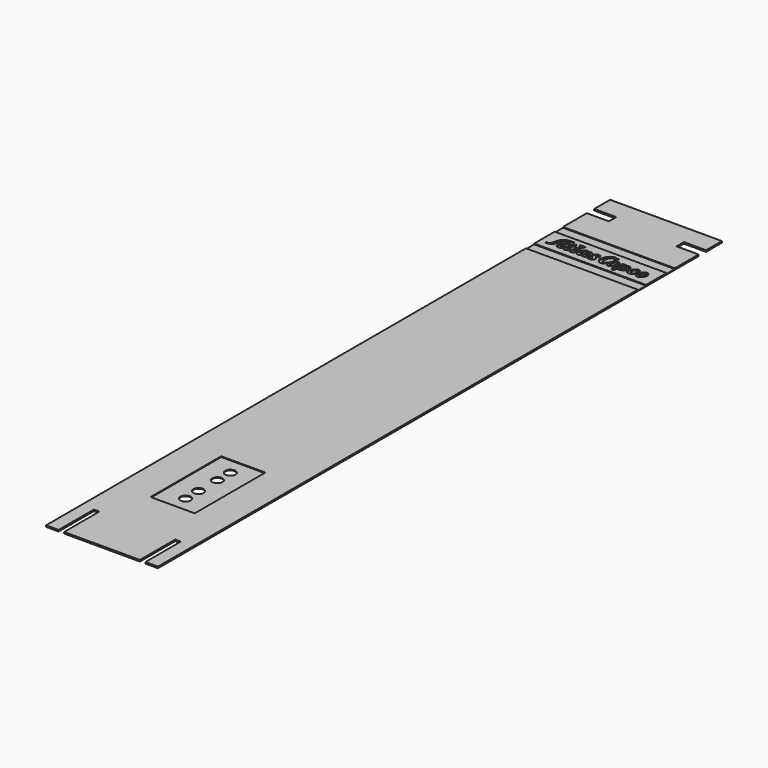
from build123d import *

# Parameters (mm, degrees)
F0_W      = 15.2
F0_H      = 95.8
F1_DEPTH  = 0.2
F3_DEPTH  = 0.2
F4_W      = 15.2
F4_H      = 1.4
F5_DEPTH  = 0.1
F6_W      = 0.75
F6_H      = 6
F7_DEPTH  = 0.2
F8_W      = 6
F8_H      = 12
F9_DEPTH  = 0.1
F10_R     = 0.7
F11_DEPTH = 0.1


# Not quite as in the source:
# - ends of sketch curves that miss each other by under 0.0002 mm in the source are joined


with BuildPart() as f1:
    # F0 (on Top) → F1 (new body)
    with BuildSketch(Plane.XY):
        with Locations((-42.5382462929, 16.9697062761)):
            Rectangle(F0_W, F0_H)
    extrude(amount=F1_DEPTH)

    # F2 (on face) → F3 (cut)
    with BuildSketch(Plane.XY.offset(0.2)):
        Polygon((-47.4382462929, 62.1697062761), (-50.1382462929, 62.1697062761), (-50.1382462929, 60.9197062761), (-47.4382462929, 60.9197062761), (-47.1382462929, 60.9197062761), (-47.1382462929, 61.2197062761), (-47.1382462929, 61.8697062761), (-47.1382462929, 62.1697062761), align=None)
        Polygon((-34.9382462929, 60.9197062761), (-34.9382462929, 62.1697062761), (-37.6382462929, 62.1697062761), (-37.9382462929, 62.1697062761), (-37.9382462929, 61.8697062761), (-37.9382462929, 61.2197062761), (-37.9382462929, 60.9197062761), (-37.6382462929, 60.9197062761), align=None)
    extrude(amount=-F3_DEPTH, mode=Mode.SUBTRACT)

    # F4 (on face) → F5 (cut)
    with BuildSketch(Plane.XY.offset(0.2)):
        with BuildLine():
            add(Edge.make_bspline(
                [(-48.7138666213, 53.7292808294), (-48.7156503517, 53.6955485624), (-48.716016697, 53.6346363779), (-48.7086367188, 53.6136479849), (-48.751245686, 53.5463738081), (-48.7435802903, 53.4949609673), (-48.7714375819, 53.457075765), (-48.7565093617, 53.4004759858), (-48.7859861913, 53.3621716148), (-48.803870122, 53.3295657915), (-48.8005908459, 53.2827188253), (-48.8191713931, 53.249915498), (-48.838998348, 53.2225362715), (-48.8612462779, 53.1887474059), (-48.9028095806, 53.1617157571), (-48.920007553, 53.1259647414), (-48.9371818267, 53.1133580395), (-48.9536866203, 53.0882073737), (-48.9963642851, 53.0676081291), (-49.0282974801, 53.065839452), (-49.0504280389, 53.0486706861), (-49.084192329, 53.0400553041), (-49.1097692251, 53.034060091), (-49.1323162662, 53.0468093828), (-49.1793725448, 53.0441402698), (-49.2251702673, 53.0557072606), (-49.247223991, 53.0507750388), (-49.2595791196, 53.069044863), (-49.3088733908, 53.0697208771), (-49.3069164004, 53.0876727693), (-49.3417040682, 53.083148655), (-49.3366722706, 53.0764487725), (-49.3388458473, 53.0493512936), (-49.3380585585, 53.0230725834), (-49.338282842, 52.9842419724), (-49.3382643659, 52.9585925934), (-49.3381407997, 52.9218855534), (-49.3385027946, 52.9121269514), (-49.3373427559, 52.889278378), (-49.3407043101, 52.8854054963), (-49.2663032152, 52.8869751081), (-49.2305385994, 52.8760277457), (-49.2134464788, 52.8752483861), (-49.1668497463, 52.8772737892), (-49.1224171734, 52.885461746), (-49.0481792536, 52.8895621616), (-49.0128983363, 52.895449458), (-48.946318944, 52.902681564), (-48.8804121351, 52.9147360177), (-48.8380581134, 52.9391134555), (-48.8009364576, 52.9491753792), (-48.756843304, 52.9705534856), (-48.7322052227, 52.9950605524), (-48.7135723835, 53.0061106727), (-48.6737402553, 53.0485726041), (-48.6467907651, 53.0447391142), (-48.6272930391, 53.065149356), (-48.6114233204, 53.0743238179), (-48.594110594, 53.098747545), (-48.5602248656, 53.1217643099), (-48.5397493222, 53.1458186723), (-48.5061735537, 53.1685144713), (-48.467777957, 53.2101353665), (-48.4346412259, 53.2705879088), (-48.4136184926, 53.3059305658), (-48.3917294835, 53.3305711498), (-48.3784695495, 53.3748964171), (-48.3640823053, 53.3854508756), (-48.3523802975, 53.4135038669), (-48.351194247, 53.4374008503), (-48.3304892635, 53.4663711512), (-48.3222410517, 53.5061417839), (-48.3131478976, 53.5410788529), (-48.306359193, 53.5751486926), (-48.289217757, 53.6003378613), (-48.28457786, 53.6386225556), (-48.2686734292, 53.6763524035), (-48.2714880257, 53.7307905469), (-48.2595446833, 53.7374505003), (-48.2552759349, 53.7398308516)],
                knots=[0, 0, 0, 0, 0.0212680281, 0.0315026842, 0.05018682, 0.0659413755, 0.0801677622, 0.0962024207, 0.1109583869, 0.1242253552, 0.1389006714, 0.1521676396, 0.1648370384, 0.1786994073, 0.194141542, 0.2076256595, 0.2174546854, 0.2292506593, 0.2441990486, 0.2564638347, 0.2677983227, 0.2807433283, 0.2916768065, 0.302312449, 0.3174054259, 0.3326037369, 0.3421239137, 0.351868523, 0.3662547428, 0.3735729434, 0.3848908404, 0.3894278876, 0.4005179797, 0.4123417421, 0.4257129452, 0.4373752731, 0.4501772837, 0.4578979236, 0.4680174761, 0.470718732, 0.4887107591, 0.5029329007, 0.5116467377, 0.5261189746, 0.5415812478, 0.5601205817, 0.5735106831, 0.5912245268, 0.6094073617, 0.6244446104, 0.6380389911, 0.6533728522, 0.6659495885, 0.6764479817, 0.6926374299, 0.7036251672, 0.7146471582, 0.724022027, 0.7358174415, 0.7498373422, 0.7621202818, 0.7757886667, 0.7924138014, 0.8107072, 0.8246133116, 0.8372827104, 0.8517630584, 0.8610040521, 0.8726348309, 0.8833773794, 0.8961563446, 0.9101559133, 0.9234366258, 0.9361787279, 0.9481124511, 0.9613931637, 0.9758818198, 0.9914420681, 1, 1, 1, 1], degree=3))
            Line((-48.2552759349, 53.7398308516), (-47.8400550783, 53.7398308516))
            Line((-47.8400550783, 53.7398308516), (-47.9847863317, 53.2937496901))
            add(Edge.make_bspline(
                [(-47.9847863317, 53.2937496901), (-47.9874138399, 53.2440943997), (-47.992459728, 53.1487359796), (-47.9603690316, 53.0124799009), (-47.9001197436, 52.9839035424), (-47.8316463543, 52.9307304547), (-47.7546096834, 52.916598056), (-47.6737373447, 52.8905118125), (-47.5364112324, 52.8772495286), (-47.4155884864, 52.8868377993), (-47.3460282165, 52.9413478526), (-47.2553008163, 52.9706081857), (-47.1936635306, 53.0184458369), (-47.1228112792, 53.0686785287), (-47.101854287, 53.1315368954), (-47.051812621, 53.1308071337), (-47.0507621407, 53.0657758634), (-47.0206957299, 52.9589705326), (-46.9528171236, 52.9499516014), (-46.8997850119, 52.8765749534), (-46.787664074, 52.8793082024), (-46.6856574409, 52.8812078692), (-46.6289790533, 52.892450117), (-46.5252269363, 52.9365512722), (-46.426211123, 52.9740201967), (-46.3435888828, 53.0312177285), (-46.2807206476, 53.056488524), (-46.2712628569, 53.1000631683), (-46.2269539779, 53.0994514966), (-46.1766632762, 53.1489929306), (-46.1624011626, 53.0508267663), (-46.1631308949, 52.9951406241), (-46.1106529437, 52.9479515463), (-46.0875080606, 52.9147453726), (-45.9985153634, 52.8942301087), (-45.9361718318, 52.8607068312), (-45.8744996576, 52.9019095971), (-45.7704275582, 52.8759565225), (-45.7325535531, 52.9191483961), (-45.6585541639, 52.9259866124), (-45.6183663938, 52.9486544637), (-45.5896380757, 52.9632385406), (-45.5697281476, 53.0035934605), (-45.4858775833, 53.0204825837), (-45.4713738375, 53.0969844284), (-45.3948728342, 53.1230677687), (-45.4049880412, 53.1837241362), (-45.3522579653, 53.2090688227), (-45.2996151623, 53.2100414297), (-45.3258294957, 53.1499251228), (-45.300256811, 53.1059045738), (-45.298245664, 53.0816229028), (-45.2638684737, 53.0421422592), (-45.2081376683, 52.9788217335), (-45.1852654038, 52.9501706504), (-45.1282373443, 52.9058124034), (-45.03662767, 52.8902994021), (-44.9938759808, 52.86390556), (-44.9710227549, 52.8683774173)],
                knots=[0, 0, 0, 0, 0.026354554, 0.0506752611, 0.0675517739, 0.0872191781, 0.1059848187, 0.125723748, 0.1510680484, 0.1744721127, 0.1943296003, 0.2149633855, 0.2340868409, 0.2540259879, 0.2706332822, 0.2825954965, 0.2989347213, 0.320879896, 0.3374297369, 0.3566714445, 0.3790289346, 0.4006540035, 0.4169291347, 0.4393798919, 0.4619565404, 0.4835602628, 0.5006647879, 0.5133187561, 0.5270214092, 0.5416120869, 0.5597839907, 0.5766751743, 0.5937284846, 0.6073571258, 0.6274969065, 0.6450229239, 0.6625645626, 0.68376343, 0.6992197931, 0.7173259646, 0.7319166423, 0.7436274968, 0.7573723576, 0.7760487224, 0.7939443974, 0.8116185946, 0.8264658184, 0.8421788155, 0.8550869449, 0.870193848, 0.8852546403, 0.8954238662, 0.9107626631, 0.9305488723, 0.9437177039, 0.9613732192, 0.9822406164, 1, 1, 1, 1], degree=3))
            add(Edge.make_bspline(
                [(-44.9710227549, 52.8683774173), (-44.9448111052, 52.8654164585), (-44.8972031546, 52.8600384992), (-44.8541460275, 52.8942944555), (-44.8088346799, 52.8893828973), (-44.7737883387, 52.9113873583), (-44.7297953365, 52.9056222124), (-44.7243131366, 52.9320694267), (-44.675834093, 52.9448570868), (-44.6687562381, 52.9667196621), (-44.6345434375, 52.9825531732), (-44.608341967, 53.0038749981), (-44.6000733357, 53.0182146773), (-44.5672448778, 53.0370344732), (-44.5516181626, 53.0526895218), (-44.5253973132, 53.0280663045), (-44.5066951806, 53.0047330268), (-44.4866595975, 52.9640184043), (-44.4525912655, 52.9480406804), (-44.444198004, 52.9173442874), (-44.419352619, 52.9136605628), (-44.4037150822, 52.9011691783), (-44.3612107793, 52.8964810767), (-44.3338102513, 52.8992906586), (-44.2826628523, 52.8966833914), (-44.2444640407, 52.9037368909), (-44.2130976999, 52.890620848), (-44.1782665479, 52.9029714216), (-44.1580797502, 52.8999974536), (-44.1189381967, 52.9116196865), (-44.0810775094, 52.9376296562), (-44.0251229873, 52.9442869569), (-44.019729484, 52.9684319526), (-43.9897573039, 52.9783441083), (-43.9675811046, 52.9889512189), (-43.9353460574, 53.0178243091), (-43.9196550147, 53.030628403), (-43.8866828659, 53.0613297288), (-43.8722231108, 53.0769638939), (-43.8514288416, 53.1016695953), (-43.8279175807, 53.0690673086), (-43.8157299716, 53.0508196698), (-43.7817352753, 53.0065930092), (-43.7608710646, 52.9946758433), (-43.7450344543, 52.9771172406), (-43.7204132698, 52.9440721259), (-43.6956226666, 52.9368571462), (-43.6697930594, 52.9241011769), (-43.6500345425, 52.9136320382), (-43.6412818387, 52.9051335078), (-43.5858485908, 52.8871846661), (-43.555304496, 52.8648907542), (-43.529121104, 52.8692185862), (-43.5052249491, 52.868090128), (-43.467769658, 52.8684672938), (-43.4346647085, 52.8683147621), (-43.3865040049, 52.8685405512), (-43.350819772, 52.8678359999), (-43.3019361595, 52.870801151), (-43.2486826509, 52.859658006), (-43.2185798377, 52.8926250597), (-43.1943017921, 52.8851441265), (-43.1455636174, 52.9202600879), (-43.100679528, 52.9347881726), (-43.0681850917, 52.9578627156), (-43.048625037, 52.9778734977), (-42.9871899802, 52.9893597305), (-42.9695565468, 53.0225921461), (-42.9498325529, 53.0623440944), (-42.9019885646, 53.0932206221), (-42.8986264628, 53.1077111042), (-42.8645610368, 53.1649491019), (-42.855480126, 53.1640229248), (-42.8487211466, 53.1877651811)],
                knots=[0, 0, 0, 0, 0.0205571512, 0.0376206784, 0.0532039933, 0.0686615953, 0.0833544329, 0.0944106211, 0.1105517311, 0.1216099328, 0.1361266636, 0.1499617098, 0.1597891633, 0.1744487366, 0.1847413111, 0.1978009762, 0.2115376913, 0.2274190555, 0.2418581016, 0.2545131606, 0.2656532014, 0.2764432163, 0.2916907218, 0.3047871844, 0.3218003326, 0.3368087705, 0.3504810098, 0.364560975, 0.3753835254, 0.3901974698, 0.4071098533, 0.4242508171, 0.4350061235, 0.4477778801, 0.460213327, 0.4755960311, 0.4870384107, 0.5027546092, 0.5146669846, 0.5262374946, 0.5395091815, 0.5518752214, 0.5694819868, 0.581267709, 0.592844865, 0.6080322045, 0.6202235408, 0.6332046106, 0.6442242425, 0.6525736671, 0.6706837612, 0.6856914371, 0.6973456195, 0.7091658203, 0.7236963657, 0.7378462892, 0.7543258323, 0.7688215135, 0.7856603612, 0.8030514895, 0.8177628597, 0.8288921979, 0.846994585, 0.8640495895, 0.8787033116, 0.891482257, 0.909763258, 0.9240243632, 0.9402840314, 0.9576557182, 0.9674687077, 0.9854086834, 1, 1, 1, 1], degree=3))
            add(Edge.make_bspline(
                [(-42.8487211466, 53.1877651811), (-42.8451361427, 53.2036741418), (-42.8383454338, 53.2338088717), (-42.8242722286, 53.2695485796), (-42.8219952065, 53.3002712502), (-42.8284401884, 53.3267873097), (-42.8220707165, 53.3564384063), (-42.836105431, 53.391737246), (-42.8261379281, 53.4212655893), (-42.8531276651, 53.4501864128), (-42.8455284977, 53.4653650275), (-42.8611982255, 53.4972541963), (-42.8875269398, 53.5269657431), (-42.9229555629, 53.5443173489), (-42.9606012727, 53.5911572243), (-42.9944302167, 53.6104590068), (-43.0203824934, 53.6216280803), (-43.0591076875, 53.6307327783), (-43.0703081325, 53.6709383172), (-43.1199918437, 53.6770010404), (-43.1383803319, 53.6957128859), (-43.1487140023, 53.7121647939), (-43.1909062348, 53.7489596325), (-43.2059561639, 53.7633180948), (-43.2218775169, 53.7827819136), (-43.2401208762, 53.8159251495), (-43.2548969299, 53.8459787605), (-43.2614580317, 53.866718888), (-43.2715554491, 53.9073193319), (-43.265536949, 53.9353326451), (-43.2618710089, 53.9590493475), (-43.2479615285, 53.9826819715), (-43.2313511055, 54.0023154775), (-43.2138809444, 54.0151531189), (-43.1927436202, 54.0269213865), (-43.1728132561, 54.0290005946), (-43.1461248706, 54.0355977129), (-43.1262871692, 54.043971747), (-43.0946443671, 54.0411558518), (-43.0752567893, 54.0398394859), (-43.0673864843, 54.0238387562), (-43.0671329121, 54.0054193915), (-43.0646471032, 53.988160414), (-43.0719703281, 53.9735982413), (-43.0722850994, 53.9615547369), (-43.0782217052, 53.9459584765), (-43.0826998907, 53.9158833694), (-43.0823242674, 53.9007955852), (-43.0885434344, 53.8664178217), (-43.0757355211, 53.858404355), (-43.0721490158, 53.8452055105), (-43.0557341492, 53.8236426225), (-43.0469951597, 53.8120028274), (-43.0348581966, 53.7909314065), (-43.0210651948, 53.7829561702), (-43.0031533841, 53.7760872177), (-42.9940630528, 53.7694604023), (-42.9718018879, 53.7530178139), (-42.9560597028, 53.7498151672), (-42.9288642324, 53.7502118834), (-42.902187742, 53.7418793947), (-42.8454611237, 53.7368746061), (-42.8173215751, 53.7771122417), (-42.7982216529, 53.7757058957), (-42.7893099781, 53.7900625448), (-42.7795788169, 53.7995626104), (-42.7602040651, 53.8203044172), (-42.7458633445, 53.8305425915), (-42.7468636329, 53.8568618384), (-42.7465736864, 53.8739530661), (-42.746424675, 53.8827367127)],
                knots=[0, 0, 0, 0, 0.0199488621, 0.0377871051, 0.0535457009, 0.0683803389, 0.0840727972, 0.1014394621, 0.1170814415, 0.1338544575, 0.1446812323, 0.1612022758, 0.1794310048, 0.1975393229, 0.2197760372, 0.2376488119, 0.2530198937, 0.2703428083, 0.2876801688, 0.3071748298, 0.3213212386, 0.3342809313, 0.3556443324, 0.3691692966, 0.3831936672, 0.4011857561, 0.417734328, 0.4313504407, 0.4497497474, 0.4652601373, 0.4791962354, 0.494205365, 0.5088036515, 0.5222777758, 0.5361977657, 0.5492048704, 0.5641133407, 0.5776672504, 0.5938350032, 0.6061166999, 0.6173926494, 0.6298813047, 0.6418742043, 0.6532227997, 0.6629723232, 0.6748391501, 0.6904557716, 0.702528956, 0.7187638704, 0.728957633, 0.7394645125, 0.7542693607, 0.7657899294, 0.7795887307, 0.7912800492, 0.8035306768, 0.8135529856, 0.8283519155, 0.8401317995, 0.8546324486, 0.8702723626, 0.8912892424, 0.9104000423, 0.921914291, 0.9328991332, 0.9438839755, 0.9591475785, 0.970943162, 0.985066901, 1, 1, 1, 1], degree=3))
            add(Edge.make_bspline(
                [(-42.746424675, 53.8827367127), (-42.7418796139, 53.8940018829), (-42.73450134, 53.9122893181), (-42.7375230601, 53.9240802519), (-42.7346062582, 53.9507124997), (-42.7505722631, 53.9630653728), (-42.7418890039, 53.9881156483), (-42.7600898717, 53.9965638679), (-42.7563950854, 54.0265337816), (-42.7727820699, 54.0308057133), (-42.7735919437, 54.0454788274), (-42.7781113773, 54.0557257786), (-42.7910490929, 54.0779970828), (-42.798656171, 54.0804862618), (-42.8048649135, 54.0921942811), (-42.8112503964, 54.1027543823), (-42.8126520812, 54.1164013808), (-42.8339632572, 54.1201824826), (-42.8443183669, 54.1356920365), (-42.8510217419, 54.1367178023), (-42.8629652659, 54.1512634912), (-42.8651181183, 54.1525824751), (-42.8657494485, 54.1529692709)],
                knots=[0, 0, 0, 0, 0.0718741397, 0.1166776581, 0.1799202695, 0.2342188716, 0.2931265712, 0.3445167497, 0.4091982061, 0.4557036828, 0.5006769947, 0.546062732, 0.6095151547, 0.645154051, 0.6900225425, 0.7359792193, 0.7793959169, 0.8362969435, 0.8892709676, 0.9231785328, 0.9774718822, 1, 1, 1, 1], degree=3))
            add(Edge.make_bspline(
                [(-42.8657494485, 54.1529692709), (-42.8747793535, 54.1617230643), (-42.8910281961, 54.1774750587), (-42.9132895871, 54.1790445614), (-42.9482687194, 54.1903227405), (-42.9672852687, 54.1944470203), (-42.9811103954, 54.2084508918), (-43.0196660427, 54.2148598396), (-43.0545260486, 54.2187330917), (-43.1015229643, 54.2202452552), (-43.1692584519, 54.2268820347), (-43.1887461415, 54.2196554669), (-43.2123821911, 54.2250583638), (-43.2296898733, 54.2172779186), (-43.2600683395, 54.2243595032), (-43.2921258273, 54.2169964354), (-43.3144620798, 54.215102236), (-43.3388974912, 54.2108493955), (-43.3675424993, 54.2055877626), (-43.3873577914, 54.1969375962), (-43.4074258602, 54.1832696045), (-43.4307370317, 54.1719104503), (-43.4476399856, 54.1630080012), (-43.5358276209, 54.1024042384), (-43.5553270905, 54.0871170807), (-43.5824798531, 54.0613749861), (-43.5872636344, 54.0482984448), (-43.5996878274, 54.0340265493), (-43.631836971, 53.9955146078), (-43.6394371842, 53.9750995724), (-43.6559516052, 53.930935472), (-43.6558398934, 53.9101931498), (-43.6886617152, 53.8652530652), (-43.674253508, 53.8313575397), (-43.6775645074, 53.7966058333), (-43.6708158922, 53.7558898793), (-43.668432256, 53.7235005067), (-43.6638111322, 53.7036796861), (-43.6699351518, 53.6628619362), (-43.6441381509, 53.6458824296), (-43.6257797256, 53.6164841305), (-43.6003585751, 53.5964338832), (-43.5799425031, 53.5676651897), (-43.5661734248, 53.5533678188), (-43.5327621611, 53.5366379487), (-43.5091219536, 53.5234555312), (-43.4764913489, 53.4958356631), (-43.4597588372, 53.4839792628), (-43.4243177794, 53.4509209156), (-43.3919568879, 53.4308308384), (-43.3470342608, 53.4088605678), (-43.3197257744, 53.382838325), (-43.2904492245, 53.3502720475), (-43.2638904815, 53.3299693134), (-43.2447518088, 53.2875636986), (-43.2323348099, 53.2459139342), (-43.2265405916, 53.1995022105), (-43.2329764447, 53.1655243746), (-43.2602998952, 53.1070250662), (-43.3148751149, 53.1067144021), (-43.3341590488, 53.0628038475), (-43.4254440927, 53.0521464221), (-43.4559563164, 53.0528212738), (-43.4776661985, 53.049084633), (-43.5098248515, 53.0457015498), (-43.5327555998, 53.0547340669), (-43.5532778127, 53.064347264), (-43.5632007866, 53.065424716), (-43.602845109, 53.0616462685), (-43.6132880503, 53.0909941256), (-43.6227418699, 53.1049322609), (-43.641438095, 53.1244833079), (-43.6503433328, 53.1456478204), (-43.652560796, 53.1633580271), (-43.6643199102, 53.2001102512), (-43.6356994807, 53.2050144692), (-43.6045708054, 53.2020444659), (-43.5876405766, 53.2261480929), (-43.5750920889, 53.2238266287), (-43.5596855646, 53.2504369941), (-43.5662901952, 53.2604030649), (-43.5588219219, 53.2745328704), (-43.5595640948, 53.2932549554), (-43.5622608295, 53.3116877023), (-43.563579296, 53.3377831718), (-43.5556855501, 53.3753375114), (-43.5632507974, 53.3975301415), (-43.5714413819, 53.4207003941), (-43.5921587354, 53.4273036961), (-43.6090100176, 53.4495185906), (-43.6265928195, 53.4671741392), (-43.6982085386, 53.4856876255), (-43.7157952969, 53.4914597114), (-43.7335073948, 53.4852258861)],
                knots=[0, 0, 0, 0, 0.0116092643, 0.0209403206, 0.0329184358, 0.0415871937, 0.050018527, 0.0621995615, 0.0740248154, 0.0879727008, 0.1041997797, 0.1132156003, 0.1224791748, 0.1309445516, 0.1418479769, 0.1532521257, 0.1626216564, 0.1725038078, 0.1832000571, 0.1924098446, 0.2022465464, 0.2119524135, 0.221177746, 0.2413655611, 0.2523854142, 0.2639403191, 0.2711625486, 0.27975174, 0.2935996842, 0.3035189054, 0.3166521849, 0.3260841581, 0.3401125285, 0.3517156358, 0.3633439681, 0.3762172021, 0.3873647491, 0.396467456, 0.4085320071, 0.419066974, 0.4306356419, 0.4420949569, 0.4536627316, 0.4626122154, 0.4744179161, 0.4852267088, 0.4978527197, 0.5071780251, 0.5206438882, 0.5332958136, 0.5471017096, 0.5594459268, 0.5724150895, 0.5838748598, 0.5971366937, 0.6104862918, 0.6237558521, 0.6356519196, 0.6508098122, 0.6642646376, 0.6770999602, 0.6956104672, 0.7067509322, 0.7158388388, 0.7269806214, 0.7370328803, 0.7461242269, 0.7526358824, 0.7643495028, 0.7746335739, 0.7829357264, 0.7931599988, 0.8024847488, 0.8112690284, 0.8224172305, 0.8316634343, 0.8427934739, 0.8527057474, 0.8592450518, 0.8694578435, 0.8758949342, 0.8833836745, 0.8919513514, 0.9004667963, 0.9106776725, 0.9228755804, 0.9325511474, 0.9419288573, 0.9508739834, 0.9610012428, 0.9710734327, 0.9875159781, 1, 1, 1, 1], degree=3))
            add(Edge.make_bspline(
                [(-43.7335073948, 53.4852258861), (-43.7468010752, 53.4868585359), (-43.7704510632, 53.4897630851), (-43.784289946, 53.4704133021), (-43.8141167545, 53.4561721366), (-43.827133612, 53.4338515882), (-43.8450807084, 53.4265688511), (-43.8631627485, 53.4153225232), (-43.8666527427, 53.3993687674), (-43.8718947787, 53.3861221164), (-43.8765593824, 53.3744836743), (-43.8766544907, 53.3527995949), (-43.8782408916, 53.330783249), (-43.8725429836, 53.3136054161), (-43.8815885018, 53.2965391342), (-43.8763959265, 53.2825940846), (-43.8891361471, 53.2607229712), (-43.9003117822, 53.2468470876), (-43.9205720075, 53.2348333346), (-43.9349692158, 53.2182580468), (-43.9536311165, 53.2082583866), (-43.9709651661, 53.1815242812), (-43.9834549133, 53.1792394749), (-44.0032433606, 53.1787845738), (-44.0395079401, 53.1864969116), (-44.078912193, 53.1786067033), (-44.099844907, 53.1853180769), (-44.1216194382, 53.1933450966), (-44.1289407146, 53.2046224828), (-44.1434141275, 53.2277563586), (-44.1458078617, 53.2508485756), (-44.135138951, 53.2745486247), (-44.1382288121, 53.3144053894), (-44.123431147, 53.3410446146), (-44.1299560388, 53.3643718842), (-44.115666773, 53.3799215948), (-44.1172097673, 53.4049932435), (-44.1109720611, 53.424096756), (-44.0941703296, 53.4744723075), (-44.1048786039, 53.5038954589), (-44.092218526, 53.5236656801), (-44.0863778315, 53.5445963791), (-44.083932535, 53.5641131241), (-44.0755107559, 53.5801442218), (-44.0692372959, 53.5945505522), (-44.0625073374, 53.6240938836), (-44.0668561677, 53.6562167141), (-44.0488712049, 53.6782440571), (-44.0476727504, 53.7105914129), (-44.0422186602, 53.737710829), (-44.0363619982, 53.7559349083), (-44.0216642005, 53.8756081778), (-43.9944077593, 53.9693309257), (-43.9849243123, 54.0097515647), (-43.9594170255, 54.052130355), (-43.9648757732, 54.0800009727), (-43.9383412885, 54.1063958883), (-43.9460855544, 54.1460575306), (-43.9357877442, 54.1644018073), (-43.943332569, 54.1794126676), (-43.9644230906, 54.1695271105), (-44.0387023964, 54.1710267176), (-44.0876531345, 54.1855335127), (-44.1188139303, 54.1772846933), (-44.1641628656, 54.1730044701), (-44.1965513121, 54.1791542708), (-44.2534853761, 54.1703368579), (-44.3081872981, 54.1908809932), (-44.3132769425, 54.1223629783), (-44.3188125521, 54.0828496344), (-44.3799629735, 54.1127278323), (-44.3948852334, 54.1271943395), (-44.4021574321, 54.1475887083), (-44.4371124046, 54.1778726121), (-44.4589670466, 54.18589438), (-44.5082611171, 54.1911543616), (-44.5256035333, 54.2078197235), (-44.5922014281, 54.2072199514), (-44.6360742708, 54.2133152985), (-44.6979516103, 54.2144473628), (-44.7189958884, 54.210597081), (-44.755327422, 54.2042696508), (-44.8284936392, 54.2038465651), (-44.817176987, 54.1697821606), (-44.8493886999, 54.1623299229), (-44.8800929107, 54.1390506104), (-44.904496811, 54.1231838351), (-44.9427572702, 54.1063780397), (-44.9645042473, 54.0825245229), (-44.9894442111, 54.0614759975), (-45.0009662133, 54.0422142691), (-45.0111681185, 54.0245530517), (-45.0167022645, 54.0149733424)],
                knots=[0, 0, 0, 0, 0.0121059892, 0.0215165969, 0.0331013884, 0.0432455659, 0.052117632, 0.061253396, 0.0693129667, 0.0769241301, 0.0840664715, 0.0935091801, 0.1031748674, 0.1116655493, 0.1201577577, 0.1277052334, 0.1375972837, 0.1463770857, 0.1561239045, 0.1655652956, 0.1750819024, 0.1862568609, 0.1931491734, 0.2019515518, 0.2145022571, 0.2273231773, 0.2369177673, 0.2463595513, 0.2537884555, 0.264285912, 0.2739130339, 0.284151305, 0.2969230805, 0.3080178158, 0.3174156329, 0.3263118085, 0.3360735888, 0.3454784228, 0.3601241126, 0.3712488704, 0.3806360382, 0.3901471837, 0.3991926161, 0.4076793682, 0.4157394694, 0.4268907687, 0.4383244974, 0.4487821516, 0.4603704123, 0.4707630989, 0.4795346537, 0.5017383345, 0.5224015586, 0.5355011626, 0.5493365335, 0.5597075019, 0.5714507241, 0.5840388984, 0.5931255337, 0.5999329432, 0.6087471854, 0.6264387605, 0.6410952441, 0.6524740473, 0.6659398026, 0.677775403, 0.6933524922, 0.7068677258, 0.7221809663, 0.7331857783, 0.7483555425, 0.7579011321, 0.7671037595, 0.7806033016, 0.7909678741, 0.8047559554, 0.8147545749, 0.8307154769, 0.8452380358, 0.8608442639, 0.8701345022, 0.8829408038, 0.8990144603, 0.9082386594, 0.9188686249, 0.9316502191, 0.9428083931, 0.9557607998, 0.967498117, 0.9789316128, 0.9885612608, 1, 1, 1, 1], degree=3))
            add(Edge.make_bspline(
                [(-45.0167022645, 54.0149733424), (-45.0405451359, 53.990585669), (-45.0860049814, 53.9440870806), (-45.128145197, 53.8696378119), (-45.1637852629, 53.8381198), (-45.2134441001, 53.7223075721), (-45.2621208302, 53.675959444), (-45.278602628, 53.6402292883), (-45.2952462078, 53.5859446436), (-45.3250338092, 53.5605237839), (-45.3521231806, 53.5247272123), (-45.3631417658, 53.4859405205), (-45.3824047911, 53.4464670774), (-45.4004884957, 53.4292077871), (-45.434558213, 53.3723008002), (-45.4559853433, 53.3446918037), (-45.4658524127, 53.3274511681), (-45.4965314654, 53.3109829124), (-45.5127842272, 53.2884882116), (-45.5335580085, 53.2645018757), (-45.5421037944, 53.2279529794), (-45.5685279589, 53.2215360996), (-45.5797030882, 53.1955931587), (-45.6026797459, 53.1853357178), (-45.6181884874, 53.1720640131), (-45.6643964937, 53.1645372317), (-45.7030677208, 53.1807534948), (-45.7229913542, 53.1930602889), (-45.7324644476, 53.1967523828), (-45.7432095422, 53.2060567785), (-45.7513032579, 53.2380470613), (-45.7494369571, 53.2621392823), (-45.7287936824, 53.2918982317), (-45.7255327098, 53.3286649049), (-45.707653612, 53.3572747951), (-45.7081626241, 53.3867685019), (-45.6939958033, 53.4038673341), (-45.697232296, 53.4335739954), (-45.6864223734, 53.4456785967), (-45.6777697884, 53.4880498801), (-45.6644469801, 53.5321103021), (-45.6610103181, 53.5954003037), (-45.6302415988, 53.6225787765), (-45.6429758684, 53.663744481), (-45.6124415119, 53.7024472013), (-45.6252009304, 53.7390702771), (-45.6076142765, 53.7717751749), (-45.6022317078, 53.8319677472), (-45.591616599, 53.9052853132), (-45.5772963673, 53.9456036385), (-45.5718040466, 53.9605654776)],
                knots=[0, 0, 0, 0, 0.0338896092, 0.0640516087, 0.0874774462, 0.1247779298, 0.152340729, 0.1730876844, 0.1978719234, 0.2189335101, 0.2409766533, 0.2626866144, 0.2842744498, 0.3014635806, 0.3286933988, 0.3487327363, 0.3632593676, 0.3825761614, 0.4003848653, 0.419343154, 0.4390695091, 0.4553855783, 0.4725737469, 0.4888905317, 0.5039402934, 0.5263481508, 0.5483907918, 0.5642714996, 0.5745547483, 0.5866683392, 0.6056256659, 0.6221855581, 0.6419099945, 0.6622816493, 0.6816161069, 0.6992457019, 0.7147549327, 0.7321654789, 0.7453562944, 0.7667089086, 0.7904252688, 0.816644069, 0.8367923968, 0.8572885883, 0.8798070364, 0.8994753897, 0.9191587641, 0.9452093399, 0.9746493683, 1, 1, 1, 1], degree=3))
            add(Edge.make_bspline(
                [(-45.5718040466, 53.9605654776), (-45.5632708306, 53.9874090174), (-45.5454215685, 54.0435586479), (-45.5174180148, 54.1528502268), (-45.4989624349, 54.2236690534), (-45.4685569848, 54.3990271437), (-45.4177590003, 54.5638338402), (-45.3846480317, 54.6676417643), (-45.3507851112, 54.7593170924), (-45.5303503531, 54.7398151137), (-45.6706024387, 54.7642472373), (-45.8257548764, 54.7467732544), (-45.9501488488, 54.7555208616), (-45.9885120658, 54.7426525602), (-46.0564903893, 54.752030494), (-46.0721047707, 54.6834064248), (-46.0621782987, 54.6361268004), (-46.0700621407, 54.5796303284), (-45.9688533835, 54.5964121583), (-45.9047527135, 54.5923602985), (-45.8525055272, 54.6020308784), (-45.834299933, 54.5634287362), (-45.8477740258, 54.5132707624), (-45.8500471396, 54.4744292114), (-45.8570718765, 54.4567927718)],
                knots=[0, 0, 0, 0, 0.0466997782, 0.0985031975, 0.1414992492, 0.2071896714, 0.2737168552, 0.3267684899, 0.3653359316, 0.4242386964, 0.486654081, 0.5491540595, 0.6032995148, 0.6351469523, 0.6722511716, 0.7097668048, 0.7459860222, 0.7767604558, 0.822153374, 0.8647765128, 0.8979908744, 0.9264314043, 0.9621836785, 1, 1, 1, 1], degree=3))
            add(Edge.make_bspline(
                [(-45.8570718765, 54.4567927718), (-45.8623224611, 54.4352469816), (-45.8740765872, 54.3870138885), (-45.8939589138, 54.2848959318), (-45.9180481439, 54.1598444712), (-45.9319780244, 54.0433690316), (-45.9531487223, 53.9675791902), (-45.9790953748, 53.8839906408), (-46.0033573035, 53.7731938056), (-46.0151361201, 53.7178116622), (-46.031967498, 53.6579929221), (-46.0549579784, 53.5976100597), (-46.0802865386, 53.5605897696), (-46.0805197276, 53.5036115418), (-46.1248364608, 53.4751872476), (-46.1192239173, 53.4415887241), (-46.1655297139, 53.3974733088), (-46.1654272372, 53.3783498784), (-46.1956550162, 53.3485077948), (-46.2151504614, 53.3251862908), (-46.2590343279, 53.2907824332), (-46.2808760049, 53.2625544555), (-46.3197598169, 53.2487105373), (-46.3646674599, 53.2145104318), (-46.3923257292, 53.192573463), (-46.4376926409, 53.1793342578), (-46.4588921531, 53.1633767404), (-46.4778389391, 53.1601026529), (-46.5197595379, 53.1527582664), (-46.5468222343, 53.1459464859), (-46.5792180301, 53.1583446712), (-46.6165513793, 53.1788906631), (-46.6396001993, 53.1994365654), (-46.6497686385, 53.2362908123), (-46.6510732247, 53.286124021), (-46.6528506928, 53.3457704106), (-46.6336094315, 53.3793315497), (-46.6314917515, 53.4073174468), (-46.6149254941, 53.4370871797), (-46.6091140284, 53.4587618137), (-46.6020399477, 53.4898094805), (-46.5871191331, 53.5128407949), (-46.5826103604, 53.550395927), (-46.5860118903, 53.5892100512), (-46.5569200784, 53.6306696283), (-46.5613121158, 53.6787520344), (-46.5483795577, 53.7057925969), (-46.5566914917, 53.7549364607), (-46.5267628241, 53.7826187156), (-46.5293014443, 53.8293797893), (-46.5117396597, 53.8607273408), (-46.5167741312, 53.8922483154), (-46.5033043755, 53.9078026127), (-46.5012322666, 53.9496318828), (-46.4842832814, 53.9809433684), (-46.4947112049, 54.0369298517), (-46.4122168207, 54.0232080801), (-46.3837988087, 54.0294317046), (-46.3352803669, 54.0297727442), (-46.3119549691, 54.0281647477), (-46.2640161031, 54.024357751), (-46.2401175391, 54.0217201079), (-46.2001693514, 54.0276602448), (-46.194312327, 54.0295317125), (-46.1756156507, 54.0257001016), (-46.18007215, 54.0698903296), (-46.1779109362, 54.1071437719), (-46.1687113429, 54.1465832567), (-46.1749424916, 54.164668746), (-46.169657869, 54.1827234881), (-46.2174114517, 54.1815062053), (-46.2641467051, 54.1833384923), (-46.3310127896, 54.179941642), (-46.3957590138, 54.1969459618), (-46.4572476495, 54.1674854713), (-46.429700947, 54.2440967464), (-46.4083210435, 54.2961742506), (-46.378166188, 54.3869290969), (-46.3794289862, 54.4548255496), (-46.3650387845, 54.5195404512), (-46.34747856, 54.5578471), (-46.3952756047, 54.5850612384), (-46.4546711825, 54.5814488015), (-46.4996986835, 54.5711655369), (-46.5203779187, 54.5449215998), (-46.539483452, 54.4918091352), (-46.5446854036, 54.45565284), (-46.567554702, 54.430378699), (-46.5833799458, 54.3986114046), (-46.5923212469, 54.3820150197)],
                knots=[0, 0, 0, 0, 0.014557833, 0.0322872197, 0.0522312035, 0.071048729, 0.0862928711, 0.1027300645, 0.1212196778, 0.1343933923, 0.1480105905, 0.1619680624, 0.1735759197, 0.186232892, 0.1979132371, 0.2075416872, 0.2208394908, 0.228425906, 0.239207116, 0.2492797352, 0.2620947254, 0.2724404714, 0.2834642592, 0.2964601816, 0.3070185368, 0.3188293104, 0.3275826178, 0.3351390837, 0.3464326499, 0.355642263, 0.3656707212, 0.3770947425, 0.3865764805, 0.3969719523, 0.4094737892, 0.4228899995, 0.433458592, 0.4425930659, 0.452552392, 0.4609331731, 0.4705621866, 0.4796873842, 0.49020096, 0.5009613156, 0.5130847851, 0.5248385006, 0.5343331445, 0.5460271046, 0.5566532861, 0.5681873539, 0.5786107643, 0.5879109128, 0.5954980124, 0.6064256466, 0.6171592234, 0.6280867596, 0.6421638061, 0.6524656633, 0.6640748824, 0.6729511213, 0.6846452918, 0.6939048785, 0.7045389581, 0.7091444117, 0.7150889237, 0.7255213346, 0.7369116573, 0.7477473283, 0.7552788708, 0.7612333536, 0.7720087895, 0.7845209068, 0.798642698, 0.8133233592, 0.8246021936, 0.8374274511, 0.8516085524, 0.8682858424, 0.882905185, 0.8970412551, 0.9072250449, 0.9187557374, 0.9324751259, 0.9439632455, 0.9537324954, 0.9667784371, 0.977208925, 0.9870955427, 1, 1, 1, 1], degree=3))
            add(Edge.make_bspline(
                [(-46.5923212469, 54.3820150197), (-46.6010779122, 54.3675230913), (-46.6173203056, 54.3406425844), (-46.6527440212, 54.3297383262), (-46.6731615961, 54.2910890545), (-46.7041295491, 54.2751515923), (-46.7226788524, 54.2500932266), (-46.7342296138, 54.2309340014), (-46.7578519534, 54.2225828084), (-46.7994790494, 54.2062453266), (-46.844912011, 54.2016081163), (-46.8617269146, 54.1911744284), (-46.9136845278, 54.1986703842), (-46.9467264688, 54.1962479897), (-46.9936693849, 54.1980440708), (-47.0406973304, 54.1939402206), (-47.0831088866, 54.2115747563), (-47.0751062314, 54.1415426433), (-47.0803443194, 54.0794967607), (-47.0876859331, 54.0476874204), (-47.0879923042, 54.0275973913), (-47.0460457228, 54.0421175663), (-47.0155398319, 54.0266564729), (-46.9714223688, 54.0255660902), (-46.9359976822, 54.0195943248), (-46.912290428, 54.0260599857), (-46.8882815819, 54.023673803), (-46.8634946624, 53.996045787), (-46.8804802477, 53.9701857719), (-46.8939307767, 53.945242724), (-46.9149726437, 53.9129169589), (-46.9070508544, 53.8761225148), (-46.9257743859, 53.8484197632), (-46.9257663231, 53.8299228598), (-46.9473544549, 53.7936408318), (-46.9567196846, 53.7293678428), (-46.9635450155, 53.6725932714), (-46.9970447478, 53.6343293392), (-46.9870451838, 53.5853612657), (-47.0276446958, 53.5334594538), (-47.0391612433, 53.4873511972), (-47.061676287, 53.4569380303), (-47.0745414758, 53.397349766), (-47.1177696492, 53.344557418), (-47.1546515146, 53.2881732891), (-47.1844252296, 53.2498758683), (-47.214947693, 53.2073896669), (-47.2528554756, 53.183309431), (-47.2769027297, 53.1593331952), (-47.3197169778, 53.1363434402), (-47.3425378769, 53.1323143064), (-47.3887241293, 53.1172365806), (-47.4302601704, 53.1196458028), (-47.4788825685, 53.1240537664), (-47.5285087425, 53.1415329391), (-47.5329175513, 53.1634739155), (-47.5365913783, 53.1922054171), (-47.549510939, 53.2270278342), (-47.5267510214, 53.2843811514), (-47.5253206034, 53.3115808538), (-47.5174799821, 53.3739751148), (-47.4919763695, 53.4272502011), (-47.4854852329, 53.4809886944), (-47.4770138026, 53.5497330341), (-47.450027551, 53.632038604), (-47.4395475817, 53.6746296276), (-47.4347211421, 53.6942444742)],
                knots=[0, 0, 0, 0, 0.0167523413, 0.0310439752, 0.0466318338, 0.0609524538, 0.0743958594, 0.0855572612, 0.0973297786, 0.1139488202, 0.1301480167, 0.14087118, 0.1579449102, 0.1724499037, 0.1889387241, 0.2062252114, 0.2195374587, 0.2374756415, 0.2577119903, 0.2715627694, 0.2799501089, 0.2944150589, 0.3089476156, 0.3250424241, 0.3396364958, 0.3514461649, 0.3631570348, 0.3766803383, 0.3892281391, 0.40250197, 0.4172501901, 0.4318579095, 0.4453223842, 0.4554661962, 0.4707954417, 0.4906874316, 0.5091190426, 0.5256433632, 0.5419963381, 0.5613797735, 0.5780524505, 0.5927314798, 0.6113641072, 0.6316682884, 0.651619749, 0.6686623941, 0.6861589469, 0.7022334365, 0.7166927053, 0.7332157803, 0.7452512254, 0.7618001188, 0.7776346897, 0.7950278151, 0.8119768148, 0.822675508, 0.8355377007, 0.8503859731, 0.868922898, 0.8820297007, 0.9009316276, 0.9198273391, 0.9374830247, 0.9578171127, 0.9805551901, 1, 1, 1, 1], degree=3))
            add(Edge.make_bspline(
                [(-47.4347211421, 53.6942444742), (-47.4240728131, 53.7274564314), (-47.4030295611, 53.7930899774), (-47.3797622441, 53.8875154448), (-47.347291476, 53.9661033347), (-47.3304740229, 54.04496003), (-47.306650231, 54.1112928344), (-47.2812016874, 54.189792018), (-47.2708779037, 54.2897336993), (-47.2504400502, 54.3639463219), (-47.2312991189, 54.467628526), (-47.2092883966, 54.5156022223), (-47.2101812768, 54.5643726576), (-47.1737362175, 54.6172718868), (-47.1874705533, 54.6555991664), (-47.1697198357, 54.6909755985), (-47.0642281487, 54.6774416885), (-46.9870144824, 54.6695620892), (-46.9149941847, 54.6837246751), (-46.8841904637, 54.6744362323), (-46.8864901091, 54.7366470215), (-46.8865538551, 54.7638655573), (-46.8892231944, 54.7941172408), (-46.8960707071, 54.8163765789), (-46.8779903561, 54.846689049), (-47.0247894618, 54.8297455542), (-47.0863124986, 54.8494068462), (-47.1915066, 54.8442146676), (-47.2892903184, 54.8492511463), (-47.3953703828, 54.8487437654), (-47.4330605325, 54.8376843995), (-47.4811494758, 54.836373191), (-47.5271139271, 54.8263282324), (-47.6037656482, 54.8289823405), (-47.6405595717, 54.822929644), (-47.7042336431, 54.8098007246), (-47.7259353608, 54.812790817), (-47.7980077332, 54.8050386726), (-47.8573909074, 54.7828301506), (-47.9106449895, 54.7594142151), (-47.9363975575, 54.7573521589), (-48.0050742654, 54.7304857825), (-48.0510040152, 54.6874557054), (-48.1386816995, 54.6478296988), (-48.1721560635, 54.6190764594), (-48.2090158069, 54.5969289553), (-48.2405975679, 54.5585982219), (-48.3229090854, 54.4976663066), (-48.3487523913, 54.4843340527), (-48.3815456163, 54.4508407912), (-48.3889814942, 54.4126830416), (-48.4376015041, 54.3856611345), (-48.4391016592, 54.3391284012), (-48.504901176, 54.2651221079), (-48.5223673076, 54.2240789369), (-48.5368459406, 54.1585535039), (-48.5714120284, 54.0789434436), (-48.5996767366, 54.0193483557), (-48.6115497992, 53.955646341), (-48.6544390806, 53.861698344), (-48.6822904072, 53.8006821583), (-48.7147618103, 53.750640571), (-48.7138666213, 53.7292808294)],
                knots=[0, 0, 0, 0, 0.0217605227, 0.0427431836, 0.0623852848, 0.0813631681, 0.0991463881, 0.1185322419, 0.1396686704, 0.1588282637, 0.1804920254, 0.1958512441, 0.2104092571, 0.2269491889, 0.2398845364, 0.2511756137, 0.2722005005, 0.2921213776, 0.3100219454, 0.3197648299, 0.3349955754, 0.3469775401, 0.3584212384, 0.3687732808, 0.3772943489, 0.400762344, 0.4195418808, 0.4405667646, 0.4624476742, 0.4839984916, 0.4973357833, 0.5115548506, 0.52657025, 0.5448341027, 0.5586139938, 0.575149286, 0.5855051865, 0.6030708427, 0.6208267816, 0.6365021235, 0.6474332628, 0.6650283496, 0.6826435723, 0.7032259105, 0.7174867063, 0.7307775993, 0.746257918, 0.7675351446, 0.7794850275, 0.7933664204, 0.8065245509, 0.8212725438, 0.8354309619, 0.8561852869, 0.8706307087, 0.8877725245, 0.9077953184, 0.9249332591, 0.9420755488, 0.9634865523, 0.9816596117, 1, 1, 1, 1], degree=3))
        make_face()
        with BuildLine():
            add(Edge.make_bspline(
                [(-44.5647314191, 54.0162660182), (-44.5809467406, 54.0175234366), (-44.622442326, 54.0150613194), (-44.674766506, 54.0087829022), (-44.6896396306, 53.9779142937), (-44.7153363255, 53.9665324359), (-44.7312824362, 53.9285119314), (-44.7687098994, 53.9127114365), (-44.7816263867, 53.8399781085), (-44.8268116579, 53.8270142851), (-44.818720199, 53.7852219427), (-44.8133130152, 53.7575321626), (-44.8472044291, 53.732497077), (-44.838416472, 53.6801527288), (-44.8768007207, 53.631368763), (-44.8763568013, 53.5811267314), (-44.8910864198, 53.5422447536), (-44.9054487533, 53.5168710486), (-44.9066071425, 53.4757239896), (-44.9090899894, 53.4420539416), (-44.9092991101, 53.4090506463), (-44.9175143732, 53.3650167678), (-44.9195951122, 53.343171183), (-44.9032028503, 53.2989146229), (-44.908483375, 53.2600414492), (-44.8807327557, 53.2280659029), (-44.8715087631, 53.2041289277), (-44.8464399913, 53.1941658379), (-44.8313912861, 53.1741081107), (-44.8218919907, 53.1602090419), (-44.7583734483, 53.1652069798), (-44.7533495062, 53.1541368831), (-44.723000524, 53.1574311867), (-44.6960396268, 53.1610764129), (-44.6812271198, 53.1628577334), (-44.6424079362, 53.16820595), (-44.6362322111, 53.1794590236), (-44.6276548105, 53.2215711387), (-44.6007762047, 53.2452153251), (-44.6003944692, 53.2932729472), (-44.5804222366, 53.3189924012), (-44.5571169299, 53.3448311154), (-44.5534814643, 53.3853716386), (-44.5154384993, 53.404971439), (-44.5347399917, 53.4615333426), (-44.5061606479, 53.4722106874), (-44.4924076882, 53.4913831223), (-44.4982045675, 53.52265983), (-44.4749303931, 53.540343037), (-44.489486615, 53.5847107812), (-44.4711276527, 53.6210997462), (-44.4719951181, 53.6503497744), (-44.4476894916, 53.695008632), (-44.4612925644, 53.7278455236), (-44.4489494462, 53.7408533707), (-44.4626788315, 53.8001359133), (-44.4452888312, 53.8272083468), (-44.4515983088, 53.871250474), (-44.4409830322, 53.8992684781), (-44.4456423088, 53.9170961797), (-44.4470128035, 53.9386054757), (-44.4526751114, 53.9790202641), (-44.4652800772, 53.9958395537), (-44.5116993754, 54.0238745466), (-44.5365698396, 54.0113227994), (-44.5534663824, 54.0153924699), (-44.5647314191, 54.0162660182)],
                knots=[0, 0, 0, 0, 0.0206180881, 0.0397570311, 0.0544795489, 0.068340755, 0.0849060124, 0.1015543214, 0.1236190225, 0.1402394469, 0.1563226727, 0.1701911526, 0.1861429326, 0.2048945417, 0.2256354148, 0.2446214601, 0.2617014378, 0.2761881762, 0.2932464855, 0.3089633889, 0.3246812007, 0.342449221, 0.3552410371, 0.3732915121, 0.3901299548, 0.4070954037, 0.4205020481, 0.4340934591, 0.4472291933, 0.4580770916, 0.4786799013, 0.4871798745, 0.5014100871, 0.5156178369, 0.5266222913, 0.5428565498, 0.5521588876, 0.5692393707, 0.5854024621, 0.6033407108, 0.6185920607, 0.6342646983, 0.6508001632, 0.666911908, 0.6855487932, 0.6987887478, 0.7114109939, 0.7258057602, 0.7390516074, 0.7565098195, 0.7733507313, 0.7879244338, 0.8067865483, 0.8217112146, 0.832184426, 0.8523307183, 0.8677671007, 0.8852929306, 0.8998666331, 0.9108890696, 0.9236174666, 0.9404662111, 0.9531902536, 0.9721974023, 0.9856762927, 1, 1, 1, 1], degree=3))
        make_face(mode=Mode.SUBTRACT)
        with BuildLine():
            add(Edge.make_bspline(
                [(-48.2044927776, 53.8984574378), (-48.1600265522, 53.8574377057), (-47.8139671831, 53.8867204212), (-47.7868155747, 53.8872100223), (-47.769529589, 53.9437601259), (-47.771465791, 53.9650687512), (-47.7522947303, 54.0085372461), (-47.7528818143, 54.0405159325), (-47.7230843305, 54.1457639549), (-47.717887423, 54.2211626028), (-47.6900504889, 54.2415202952), (-47.6780998511, 54.2775150027), (-47.6679042037, 54.3253906061), (-47.652585012, 54.3502180177), (-47.6430241097, 54.4066080407), (-47.6333659177, 54.4369644626), (-47.6013894735, 54.5026292435), (-47.6061166124, 54.5376243349), (-47.5966739196, 54.5637676083), (-47.5646530255, 54.6258044833), (-47.5734650238, 54.6336028705), (-47.5641407078, 54.6902542482), (-47.6028898403, 54.6755794809), (-47.6275259303, 54.6798057676), (-47.6677166849, 54.6764921986), (-47.7067344381, 54.6859851994), (-47.7631012816, 54.6508978163), (-47.7843861628, 54.6583977228), (-47.8004770899, 54.6260482025), (-47.862022919, 54.6162548767), (-47.8694850407, 54.5710069558), (-47.9206778045, 54.5567643851), (-47.9228328408, 54.5350885544), (-47.9647915087, 54.5005465186), (-47.9824016924, 54.4635648525), (-48.0213355702, 54.4300182579), (-48.0252583366, 54.3999856442), (-48.057442997, 54.3820105897), (-48.0518006851, 54.3390286088), (-48.0814237401, 54.3212533417), (-48.0797853974, 54.2881047208), (-48.1172213942, 54.2597836234), (-48.1183138188, 54.2199213391), (-48.1448151723, 54.1698828021), (-48.1686464969, 54.1363817321), (-48.1716535044, 54.0981363936), (-48.1877999345, 54.0465060559), (-48.1873851875, 54.0086611149), (-48.2000362478, 53.9727662019), (-48.1972988324, 53.9533546075), (-48.2211179841, 53.9137940559), (-48.2044927776, 53.8984574378)],
                knots=[0, 0, 0, 0, 0.0610615639, 0.0789070293, 0.1006879231, 0.1160435541, 0.1362999384, 0.1543596989, 0.1869054367, 0.2138153355, 0.2306678324, 0.2496223639, 0.2711343244, 0.2883163345, 0.3110349245, 0.3296428799, 0.3557134526, 0.3735860072, 0.3906334371, 0.4155538003, 0.4262285835, 0.4464817344, 0.4625968069, 0.478807664, 0.498022741, 0.5179569872, 0.5424201359, 0.5554717959, 0.5724022447, 0.5956773676, 0.6153238018, 0.6361910363, 0.6497448711, 0.671844089, 0.6924966048, 0.7141046859, 0.7305554898, 0.7480158514, 0.7670441216, 0.7838964373, 0.8006957832, 0.8208372567, 0.8401361608, 0.8633997122, 0.8831535228, 0.9021825219, 0.9249012901, 0.944431929, 0.9627382361, 0.9771700633, 1, 1, 1, 1], degree=3))
        make_face(mode=Mode.SUBTRACT)
        with Locations((-42.5382462929, 56.1697062761)):
            Rectangle(F4_W, F4_H)
        with Locations((-42.5382462929, 51.2777062761)):
            Rectangle(F4_W, F4_H)
        with BuildLine():
            add(Edge.make_bspline(
                [(-41.9888794422, 54.6054206789), (-41.9978873315, 54.5976425123), (-42.0143944161, 54.583388912), (-42.0322657174, 54.5650576657), (-42.0423476645, 54.5466673455), (-42.0647355957, 54.5417245415), (-42.0700268586, 54.5087188633), (-42.0940686924, 54.4954654573), (-42.102585027, 54.4874656697), (-42.1095048664, 54.4731379924), (-42.133763561, 54.4442356612), (-42.1550713007, 54.4215108012), (-42.1797568545, 54.3931366487), (-42.1908664965, 54.3599066606), (-42.2489221726, 54.3165483963), (-42.2439023493, 54.2724444351), (-42.2663195276, 54.2276814614), (-42.2910102493, 54.2096440515), (-42.2967022106, 54.1740340398), (-42.3054247634, 54.1441701958), (-42.3147703093, 54.122819184), (-42.3309749241, 54.080966807), (-42.3364535061, 54.0623420266), (-42.3592553694, 54.0314455814), (-42.3712991534, 54.0058899431), (-42.3740492921, 53.9779853981), (-42.3864942123, 53.9536875067), (-42.3763933894, 53.9069137854), (-42.3972670662, 53.9012668488), (-42.3958006578, 53.8709652542), (-42.3990852129, 53.8538204994), (-42.4071820973, 53.8410888012), (-42.4073922206, 53.7939012882), (-42.4151841071, 53.7719654481), (-42.4171892827, 53.7397289862), (-42.4276169746, 53.6701647831), (-42.4227617313, 53.6453898884), (-42.4259028602, 53.5963739906), (-42.431782072, 53.5688845002), (-42.4331168387, 53.5082151546), (-42.4267628004, 53.4677349621), (-42.4332879631, 53.417478789), (-42.4144111422, 53.3675528065), (-42.40647874, 53.3216879281), (-42.3782687244, 53.271420824), (-42.3601504484, 53.2272301368), (-42.3497495959, 53.179508006), (-42.3242810385, 53.132445067), (-42.303462585, 53.1063268428), (-42.2816330834, 53.0690953796), (-42.2786638564, 53.0736828199), (-42.2405856157, 53.0442806631), (-42.2316073747, 53.0191557316), (-42.2051773931, 53.0053146213), (-42.1925969422, 52.9973059893)],
                knots=[0, 0, 0, 0, 0.0194880448, 0.0362928769, 0.0510221645, 0.0657005733, 0.0840020486, 0.100956594, 0.1119712139, 0.1249005437, 0.1452192832, 0.1643599309, 0.1841498741, 0.2040285076, 0.2310974712, 0.2526853785, 0.2755427987, 0.2936131851, 0.3131098798, 0.3315199445, 0.3480258071, 0.3699033934, 0.3851093883, 0.4052748305, 0.423243503, 0.4403100407, 0.4580563904, 0.4795621037, 0.4926067068, 0.5100293356, 0.5238949254, 0.5366173932, 0.5591139639, 0.5752864571, 0.5942783536, 0.6218740059, 0.6394718383, 0.6618778442, 0.6803348133, 0.7057231028, 0.7274957753, 0.7507242374, 0.774818074, 0.7976095546, 0.8226595813, 0.8457160791, 0.8690368489, 0.8928725513, 0.9137807658, 0.9338976543, 0.9383770064, 0.9600373783, 0.9783046154, 1, 1, 1, 1], degree=3))
            add(Edge.make_bspline(
                [(-42.1925969422, 52.9973059893), (-42.1615805004, 52.9840920398), (-42.10571404, 52.9602914948), (-42.0636850387, 52.9162808414), (-41.9617754698, 52.9147942969), (-41.9177521822, 52.9089774167), (-41.8689248296, 52.9109694393), (-41.8312032034, 52.9149865055), (-41.7951601549, 52.9272834752), (-41.7256489288, 52.8988395143), (-41.6904067597, 52.9352485654), (-41.6453799907, 52.9358356153), (-41.6095680025, 52.9640114551), (-41.5575652623, 52.9601356931), (-41.5198612365, 53.013316545), (-41.4924126867, 53.0178256136), (-41.4376988574, 53.0516153853), (-41.4222434681, 53.0626712341), (-41.3934546258, 53.0807174073), (-41.3685560766, 53.1018065878), (-41.3403000354, 53.1364288089), (-41.3105347267, 53.1609031554), (-41.2766937214, 53.1945534011), (-41.26435113, 53.2063098584), (-41.2592552602, 53.2111637294)],
                knots=[0, 0, 0, 0, 0.0647485678, 0.1162342244, 0.1816709035, 0.2277105616, 0.273451243, 0.3142960905, 0.3551389151, 0.4101196118, 0.454723195, 0.4981383924, 0.541968304, 0.5885342422, 0.6392252595, 0.6756439589, 0.7278869509, 0.7585433185, 0.7960889342, 0.8350445615, 0.8791153345, 0.9216701467, 0.967555755, 1, 1, 1, 1], degree=3))
            add(Edge.make_bspline(
                [(-41.2592552602, 53.2111637294), (-41.2525659509, 53.2071275264), (-41.2366474229, 53.1975225867), (-41.2388219752, 53.1515428934), (-41.2310048702, 53.1291125222), (-41.2097029084, 53.1172852021), (-41.196293085, 53.0882936661), (-41.1838808348, 53.061061993), (-41.1645619577, 53.0534051029), (-41.1356435814, 53.0128589708), (-41.1198534625, 53.0073082167), (-41.1032084259, 52.9906565593), (-41.0839392545, 52.972386106), (-41.0614408326, 52.9606932556), (-41.0503849717, 52.9413521015), (-41.0240032408, 52.9366487475), (-41.0095193349, 52.9286444608), (-40.9803342243, 52.924500181), (-40.969847606, 52.9181420318), (-40.9513525665, 52.909898422)],
                knots=[0, 0, 0, 0, 0.055817867, 0.1313770493, 0.1863095206, 0.2403442453, 0.3055241036, 0.3664002788, 0.4187721538, 0.4979083264, 0.5451772385, 0.5992180186, 0.6592574742, 0.7163609659, 0.7689277092, 0.8259900235, 0.8738411765, 0.9310132665, 1, 1, 1, 1], degree=3))
            add(Edge.make_bspline(
                [(-40.9513525665, 52.909898422), (-40.9364485097, 52.9065521813), (-40.9073446109, 52.8999978658), (-40.8664754296, 52.8865446749), (-40.8349666276, 52.8955308395), (-40.8042898097, 52.8957632817), (-40.7715934646, 52.8956100181), (-40.7410261816, 52.9132915778), (-40.7159268069, 52.9085648218), (-40.6813758854, 52.9113836663), (-40.6628115848, 52.9065635175), (-40.6502993952, 52.9243283951), (-40.6189671467, 52.9236241944), (-40.6048114374, 52.9360919869), (-40.5869714034, 52.9463821361), (-40.5575742488, 52.9577173271), (-40.5525313383, 52.9679776006), (-40.5085070684, 52.9786261358), (-40.4924164408, 53.0018599158), (-40.4503716725, 53.0093239332), (-40.4223407458, 53.0350996548), (-40.3978018079, 53.0482290028), (-40.3777361462, 53.0575989551), (-40.3506533389, 53.0791210877), (-40.3319330559, 53.0862296411), (-40.298780386, 53.1053636105), (-40.2802309358, 53.1292477094), (-40.2402675967, 53.1436469686), (-40.2320437054, 53.1768546536), (-40.1932076052, 53.1850552833), (-40.1843020981, 53.2200217815), (-40.157980701, 53.223643971), (-40.1404619615, 53.2604203296), (-40.0890785053, 53.2956552508), (-40.0667070312, 53.307696261), (-40.0363862347, 53.3616385806), (-40.0105101837, 53.3762549056), (-39.991757539, 53.3999984105), (-39.9575971657, 53.4138537761), (-39.9454556554, 53.4503966492), (-39.9191858934, 53.4519186785), (-39.9062884953, 53.4670040977), (-39.8958807811, 53.4419958641), (-39.8940348989, 53.4285113747), (-39.9030066093, 53.4064994205), (-39.9062119041, 53.3726673104), (-39.9075986411, 53.3475850111), (-39.9076313256, 53.3235033861), (-39.9170287143, 53.2965369844), (-39.9104810227, 53.2648219327), (-39.9323506304, 53.2456610442), (-39.9277019501, 53.2057126573), (-39.9461010903, 53.1819662537), (-39.9523277661, 53.1409137859), (-39.9668546529, 53.1042766653), (-39.9782064033, 53.0685045475), (-39.9831994377, 53.0191786801), (-39.9914448186, 52.9929801431), (-40.0053703627, 52.9436458671), (-39.9992510563, 52.9102984295), (-40.0178023544, 52.8779979687), (-40.0231243588, 52.8557792145), (-40.0246444606, 52.8317940187), (-40.0374983273, 52.7998127179), (-40.0355813116, 52.7836429025), (-40.0346956589, 52.776340401)],
                knots=[0, 0, 0, 0, 0.0195450247, 0.038205936, 0.0543979054, 0.0702986383, 0.0867861082, 0.1033779234, 0.1179337323, 0.1348999475, 0.1467851508, 0.1591322744, 0.1747473991, 0.186950683, 0.2003557803, 0.2160725402, 0.2256844431, 0.2442065877, 0.2595946047, 0.2777899226, 0.2956646154, 0.3106104176, 0.3243479718, 0.3409530324, 0.3542228117, 0.37159904, 0.3877518513, 0.4057462398, 0.4215623065, 0.4385590317, 0.4546074804, 0.4680120062, 0.486070588, 0.5085072715, 0.5235838794, 0.5455881713, 0.5614561452, 0.5768688255, 0.5940862438, 0.6109561906, 0.6250344317, 0.6355231293, 0.6485510628, 0.6595741807, 0.6732849175, 0.6902367728, 0.7047873505, 0.7187379901, 0.7341381923, 0.7498244481, 0.7644324962, 0.7818741684, 0.7974552349, 0.8158136275, 0.8339275296, 0.8518427041, 0.8717789797, 0.8873686039, 0.9075885994, 0.9244591343, 0.9415264294, 0.9552371662, 0.9693331545, 0.9861262001, 1, 1, 1, 1], degree=3))
            add(Edge.make_bspline(
                [(-40.0346956589, 52.776340401), (-40.0426353751, 52.7647700322), (-40.0564219234, 52.7444561364), (-40.0538957407, 52.719471085), (-40.0568042471, 52.6956433536), (-40.0657103063, 52.6776639501), (-40.0667128129, 52.6480582999), (-40.0744067951, 52.6247736912), (-40.0766257757, 52.5998968757), (-40.0885472629, 52.5806441644), (-40.0937790365, 52.5401023949), (-40.0962189234, 52.5289026946), (-40.1189703569, 52.4813604312), (-40.0681322812, 52.4788636014), (-40.0365136211, 52.4821829753), (-39.9895758985, 52.4850539109), (-39.9651474335, 52.4818130068), (-39.8963773584, 52.4739510743), (-39.8735634308, 52.4722571953), (-39.8412777709, 52.4793961756), (-39.8223687653, 52.4734918187), (-39.7803957493, 52.4696579316), (-39.771205088, 52.4681555708), (-39.7561580189, 52.471648542), (-39.7402937938, 52.4838849526), (-39.7263580067, 52.5013504706), (-39.7280605541, 52.5254555623), (-39.7098880408, 52.5568234399), (-39.7093588277, 52.6010584346), (-39.7018203315, 52.6343070551), (-39.6947848553, 52.6927947758), (-39.682081952, 52.7115716346), (-39.6726486301, 52.7566550273), (-39.6644180701, 52.7745880874), (-39.6619084238, 52.8167165262), (-39.6564525853, 52.83587902), (-39.6557169783, 52.8654001752), (-39.6447541173, 52.9097073255), (-39.6343940372, 52.9437346113), (-39.6258373469, 52.9657825602), (-39.6215314891, 52.9910330629), (-39.6071934499, 52.9978838636), (-39.598876494, 52.9976020043), (-39.5880850448, 53.0002638698)],
                knots=[0, 0, 0, 0, 0.028042631, 0.0503146672, 0.0721202906, 0.0924289934, 0.116824364, 0.1396293794, 0.1616140401, 0.1837570579, 0.2118123479, 0.2293447207, 0.2575049141, 0.2846661876, 0.3123118209, 0.3422765948, 0.3662651498, 0.4032966829, 0.4263026187, 0.4509529959, 0.4723475907, 0.5012408608, 0.515441058, 0.5323617224, 0.552865201, 0.5736986319, 0.5952361149, 0.6222779918, 0.6519469024, 0.6795329926, 0.7134481854, 0.7360268482, 0.765715797, 0.7871145512, 0.8158122915, 0.8364060715, 0.8605541293, 0.8916149819, 0.9187573766, 0.9411171222, 0.9633229211, 0.9793227824, 1, 1, 1, 1], degree=3))
            add(Edge.make_bspline(
                [(-39.5880850448, 53.0002638698), (-39.5811487754, 52.9946502268), (-39.565809949, 52.9896658911), (-39.5490119542, 52.9707507038), (-39.5359218807, 52.9670238457), (-39.5207262627, 52.9575109776), (-39.5125168053, 52.9476412505), (-39.4939058229, 52.9428317228), (-39.4915775488, 52.9404846698), (-39.4854041717, 52.9316939646), (-39.4742668417, 52.9320008371), (-39.4648242808, 52.9244131119), (-39.4551833272, 52.9238298189), (-39.449906281, 52.9188330049), (-39.4255281572, 52.9217162927), (-39.4119337886, 52.9167307185), (-39.3949256181, 52.9193565241), (-39.3550931637, 52.9163186871), (-39.3288835994, 52.9061134916), (-39.2892009087, 52.9173079883), (-39.2707811654, 52.9100487919), (-39.2242564168, 52.9181593851), (-39.1982123793, 52.9240976535), (-39.1831162326, 52.9273815658), (-39.1397700326, 52.9460659037), (-39.1184292658, 52.9572233346), (-39.0951775943, 52.9632844781), (-39.0587067307, 52.9801688295), (-39.023796193, 53.0055249714), (-39.0035661738, 52.9936650788), (-38.9799493883, 53.026109298), (-38.9754099224, 53.0371120758), (-38.9543894341, 53.0583838287), (-38.9316090306, 53.061002071), (-38.9174333797, 53.0731057768), (-38.9025881886, 53.0892051756)],
                knots=[0, 0, 0, 0, 0.0328414532, 0.0646612907, 0.0887649759, 0.1155909648, 0.1399286389, 0.1673189183, 0.1794844505, 0.1994439689, 0.2207614369, 0.2432012585, 0.262605376, 0.2793891252, 0.3108892181, 0.3357923814, 0.3623575096, 0.4031170724, 0.4387690966, 0.4787183509, 0.5080843282, 0.5524875812, 0.5861340034, 0.611935867, 0.656365095, 0.689106281, 0.7201035605, 0.7624254244, 0.8039157684, 0.8314773399, 0.8696848454, 0.894332407, 0.9283449773, 0.9578222493, 1, 1, 1, 1], degree=3))
            add(Edge.make_bspline(
                [(-38.9025881886, 53.0892051756), (-38.894830674, 53.0937165322), (-38.87761338, 53.1037291917), (-38.8406586966, 53.1279773569), (-38.8206978611, 53.149921713), (-38.7867872529, 53.1789470995), (-38.7592518539, 53.2001203362), (-38.7283025427, 53.2320010939), (-38.6941970541, 53.2577519403), (-38.6815243333, 53.2722578999), (-38.6498902664, 53.2954925442), (-38.6278084176, 53.319949589), (-38.5964004053, 53.3462766848), (-38.5711471954, 53.3719960584), (-38.5508800477, 53.3888297776), (-38.5389346326, 53.4004470025), (-38.5341233373, 53.4052202487)],
                knots=[0, 0, 0, 0, 0.0649138635, 0.1440720539, 0.2111510726, 0.2903391875, 0.3622021859, 0.443320359, 0.5210092892, 0.574435772, 0.6481450134, 0.7189098853, 0.7957521688, 0.8683740304, 0.9336386837, 0.9778533905, 0.9778533905, 0.9778533905, 0.9778533905], degree=3))
            add(Edge.make_bspline(
                [(-38.5341233373, 53.4052202487), (-38.5222735117, 53.4162997864), (-38.5024199834, 53.434901199), (-38.4846529736, 53.4475341966), (-38.4813334549, 53.4688071077), (-38.45126634, 53.4893118709), (-38.4476343703, 53.4726879622), (-38.4469044535, 53.4594796495), (-38.4432137288, 53.4393117976), (-38.4449645958, 53.4111666886), (-38.4547268279, 53.4064029247), (-38.4576224307, 53.3841199897), (-38.4636580213, 53.3653576443), (-38.4584741358, 53.3448640274), (-38.4606465108, 53.3271516279), (-38.4562006147, 53.2936991375), (-38.4505187167, 53.2632652724), (-38.4463037979, 53.2381484568), (-38.438223813, 53.2070773344), (-38.4330369245, 53.1819024897), (-38.4190840933, 53.1557932134), (-38.4029495001, 53.1279367287), (-38.3964340704, 53.1010365834), (-38.3900305946, 53.0907755101), (-38.3810905067, 53.0723095563), (-38.3638595219, 53.0574645786), (-38.3570108299, 53.0224601968), (-38.3431407092, 53.0033418131), (-38.327918025, 52.9826300655), (-38.3024211209, 52.9615219584), (-38.2774924115, 52.9536255252), (-38.2636168359, 52.9397564462), (-38.2409954171, 52.9235872383), (-38.2172045689, 52.9130900681), (-38.1653819904, 52.9073039638), (-38.1575985693, 52.8983420346), (-38.1274023178, 52.9006181938), (-38.1062611275, 52.8839118731), (-38.0609033608, 52.8829630595), (-38.0506645871, 52.8818131507), (-38.0205200459, 52.8838138942), (-38.0015290967, 52.8856125403), (-37.9567104803, 52.8804554882), (-37.9341406172, 52.8851235915), (-37.9143680579, 52.8892514346), (-37.8893073497, 52.8974601423), (-37.8683985503, 52.9011714354), (-37.8393939791, 52.9087692221), (-37.8129866752, 52.9183272542), (-37.7904773493, 52.927759216), (-37.7602295443, 52.9374772745), (-37.7364373226, 52.9558134822), (-37.7222820742, 52.9678314739), (-37.7052585973, 52.9803853801), (-37.6869518512, 52.991538231), (-37.6556296828, 52.9997450628), (-37.6384546037, 53.0222123105), (-37.6308150589, 53.0234500766)],
                knots=[0, 0, 0, 0, 0.0243573973, 0.0405882367, 0.0574765657, 0.0768756678, 0.088710957, 0.1022482651, 0.1192187802, 0.1378898175, 0.1489305894, 0.1655445513, 0.1821145247, 0.1982937366, 0.213705931, 0.234801561, 0.2552778951, 0.2737388039, 0.2942618357, 0.3127924585, 0.3324613679, 0.3535456573, 0.3723339563, 0.3849856224, 0.4009864671, 0.4183835499, 0.4397218508, 0.4574421867, 0.4758340008, 0.4968009048, 0.5151798964, 0.5311938363, 0.5498614033, 0.5694234158, 0.5950517688, 0.6073441182, 0.625966422, 0.6455288949, 0.6692173769, 0.6817981692, 0.700924607, 0.7178878524, 0.742006532, 0.7597015632, 0.7759103281, 0.7944618213, 0.8114526698, 0.8313481583, 0.8507130985, 0.8687178206, 0.8893083399, 0.9091921305, 0.9249497547, 0.9414088614, 0.9582276839, 0.9791971093, 1, 1, 1, 1], degree=3))
            add(Edge.make_bspline(
                [(-37.6308150589, 53.0234500766), (-37.6206598417, 53.0338276367), (-37.602144208, 53.055452772), (-37.5777209565, 53.0695367873), (-37.5575869481, 53.0904576182), (-37.5511012971, 53.1012155116)],
                knots=[0, 0, 0, 0, 0.3569995656, 0.6520563529, 1, 1, 1, 1], degree=3))
            add(Edge.make_bspline(
                [(-37.5511012971, 53.1012155116), (-37.5394061907, 53.1096574058), (-37.5177636194, 53.125279692), (-37.4980669125, 53.1480726904), (-37.4832334267, 53.1728888062), (-37.4660177853, 53.1911950414), (-37.4390740523, 53.2065007181), (-37.4335527314, 53.2307228409), (-37.4163431887, 53.2390201815), (-37.4077655598, 53.2534551882), (-37.3936893475, 53.2705498791), (-37.3812459163, 53.2783684203), (-37.3666775258, 53.2919814088), (-37.3582554926, 53.2981844929), (-37.341210958, 53.3039382554), (-37.344156998, 53.2802454435), (-37.3417739331, 53.2657089887), (-37.3382967187, 53.254099122), (-37.3364947145, 53.2296447796), (-37.3333765827, 53.2083707302), (-37.322276185, 53.1759702901), (-37.3198568079, 53.1448248964), (-37.3033101226, 53.1323971635), (-37.2963649005, 53.1178198206), (-37.2874026108, 53.1013211458), (-37.2794576952, 53.0836006978), (-37.2641309942, 53.0726853628), (-37.2592753052, 53.0521277913), (-37.2439187852, 53.0349155022), (-37.2311861325, 53.0276925539), (-37.2139481965, 52.9962801488), (-37.1995978333, 52.9943922455), (-37.187311959, 52.9754074399), (-37.1599816256, 52.9594639083), (-37.147735162, 52.9510208027), (-37.1293364603, 52.9350932482), (-37.1152677342, 52.9213639954), (-37.0903728212, 52.9064824651), (-37.0703502608, 52.914654932), (-37.0400484385, 52.8924813784), (-37.0214920045, 52.8926442623), (-36.9888059245, 52.8810984465), (-36.9626749904, 52.8746381551), (-36.9192255245, 52.8772035763), (-36.8962556124, 52.8751174726), (-36.8694702365, 52.8671934876), (-36.8443271709, 52.8734409526), (-36.8078911184, 52.8780024772), (-36.783794457, 52.88484083), (-36.7611813738, 52.8891934471), (-36.7272599827, 52.8924532858), (-36.6902603739, 52.8998460682), (-36.6634330954, 52.9019250902), (-36.6610974059, 52.909800108), (-36.633535326, 52.9200021356), (-36.6218565774, 52.9333768277), (-36.5919299263, 52.9541285203), (-36.5703767595, 52.9555186389), (-36.53297568, 52.9798783728), (-36.5074145438, 52.9872322377), (-36.4716309405, 53.0290049745), (-36.4574214626, 53.0259495601), (-36.432779142, 53.0583233021), (-36.419523698, 53.0697719878), (-36.4022714947, 53.0894766766), (-36.3890775244, 53.1008299642), (-36.373015435, 53.1206305293), (-36.3554554284, 53.1430025876), (-36.3434475124, 53.1506962832), (-36.3238351656, 53.1687663076), (-36.3166843689, 53.1839545927), (-36.3042517691, 53.1929166201), (-36.2972707693, 53.2142100484), (-36.281851508, 53.2232088766), (-36.2721298697, 53.2343950462), (-36.2639452826, 53.2475887424), (-36.259315908, 53.2550513744)],
                knots=[0, 0, 0, 0, 0.0181010093, 0.0334971203, 0.0484103791, 0.0625803159, 0.0778996137, 0.0913136632, 0.1029829403, 0.1145198887, 0.1275665862, 0.138600985, 0.150875227, 0.1605338461, 0.1701857235, 0.1822429286, 0.1934065017, 0.203094098, 0.2167644256, 0.230056151, 0.246561308, 0.2620629954, 0.274244565, 0.2854062236, 0.2976186961, 0.3099336393, 0.3217594711, 0.3345378565, 0.34762458, 0.358749299, 0.3749692905, 0.3851051275, 0.398091421, 0.4138217256, 0.4249441873, 0.4384282981, 0.4513617473, 0.4657865012, 0.4782881799, 0.4946584158, 0.5070302785, 0.523093461, 0.5381920912, 0.5564427908, 0.570231891, 0.5845586673, 0.5989461792, 0.6159808409, 0.6300563676, 0.6433402445, 0.6597449638, 0.6776671925, 0.6913341161, 0.6985622137, 0.7130835592, 0.7257079963, 0.742013294, 0.75540098, 0.7734849204, 0.7889519437, 0.8087732949, 0.8188702183, 0.835937109, 0.8485544096, 0.8624899503, 0.874337314, 0.8886160408, 0.9034497374, 0.9142736719, 0.9285510057, 0.940049526, 0.9507559893, 0.9637630726, 0.9753545903, 0.986060038, 1, 1, 1, 1], degree=3))
            add(Edge.make_bspline(
                [(-36.259315908, 53.2550513744), (-36.2534558599, 53.2647242789), (-36.2430826292, 53.2818468805), (-36.2377645206, 53.2987451606), (-36.2068025875, 53.3372860644), (-36.2044703707, 53.3704171624), (-36.1861425236, 53.4038285711), (-36.1796592166, 53.4576286076), (-36.1530955787, 53.510981942), (-36.1337674619, 53.5702727861), (-36.1387731912, 53.6518353235), (-36.1386944438, 53.6837916919), (-36.1335760511, 53.774805171), (-36.1512803637, 53.8498927928), (-36.1534458052, 53.8737919225), (-36.1665493349, 53.9243560685), (-36.1750837806, 53.94928209), (-36.2018717327, 53.9637332678), (-36.2057949851, 54.007742198), (-36.2371063367, 54.0304318169), (-36.2601620105, 54.0531109447), (-36.2807231017, 54.0811910818), (-36.3169717194, 54.1085556348), (-36.3261211609, 54.139605333), (-36.3520986608, 54.1552487515), (-36.386532165, 54.1681490894), (-36.4193840676, 54.190689999), (-36.4676322173, 54.1986179127), (-36.5034955605, 54.2080502453), (-36.5371999684, 54.2107694492), (-36.5859384593, 54.2078774337), (-36.622883569, 54.2019292811), (-36.6821677057, 54.1958836219), (-36.7110420285, 54.188128541), (-36.7564638252, 54.1705092112), (-36.8298232234, 54.1462709966), (-36.8590029986, 54.1159627735), (-36.9010027632, 54.0803020408), (-36.9301311945, 54.0680087797), (-36.944491185, 54.0489255596), (-36.9795457414, 54.0404602709), (-36.9903047055, 54.0250857938), (-37.0161397411, 53.9740570867), (-37.0442016794, 53.9598865806), (-37.0895818705, 53.9169307259), (-37.1193327381, 53.8820024883), (-37.1407224021, 53.8290599833), (-37.1685918318, 53.8095772632), (-37.1829936454, 53.7712194849), (-37.2033459522, 53.7482960683), (-37.2335678673, 53.7177364078), (-37.2512752893, 53.6804044225), (-37.2797208209, 53.6530087548), (-37.3072570712, 53.5950852458), (-37.3301257011, 53.5690519755), (-37.3539978616, 53.5440068868), (-37.3721023299, 53.5179784288), (-37.3973974947, 53.4932374485), (-37.4144279572, 53.4411456661), (-37.4408488809, 53.4207082559), (-37.4684814169, 53.3823332557), (-37.5010867271, 53.3577762439), (-37.5085191875, 53.3289597586), (-37.5363128236, 53.3131236229), (-37.5627845099, 53.2866639942), (-37.598748493, 53.253678063), (-37.6307715008, 53.2379577889), (-37.646188608, 53.2129809344), (-37.6745192768, 53.196964528), (-37.701165495, 53.1859936833), (-37.7122047599, 53.1718447105), (-37.7323040422, 53.161020788), (-37.7578026395, 53.1542212502), (-37.7681456665, 53.1388695602), (-37.7898856655, 53.1411607664), (-37.8112205598, 53.1317021006), (-37.8362297264, 53.124797528), (-37.8538775352, 53.1274703868), (-37.8776459411, 53.1259225061), (-37.8917757294, 53.1215725809), (-37.9030310068, 53.1288409436), (-37.9235233686, 53.1305891131), (-37.936597684, 53.1381659885), (-37.9439122443, 53.1448935911), (-37.9500420718, 53.1486234262), (-37.9531830549, 53.1505346298)],
                knots=[0, 0, 0, 0, 0.0112173729, 0.01985656, 0.0336909831, 0.0453487849, 0.0575323136, 0.0723218994, 0.0878353144, 0.1040843959, 0.1218962324, 0.1336335106, 0.1528951006, 0.1705569209, 0.1806754702, 0.1950314133, 0.2053882515, 0.2157856354, 0.2286410017, 0.2409611744, 0.2523873528, 0.2643649063, 0.2778419031, 0.2889869561, 0.2997269849, 0.3119559042, 0.3247291733, 0.3387922147, 0.3510602202, 0.3628130985, 0.3767066842, 0.3895207976, 0.4048699377, 0.4159358225, 0.4300151381, 0.4476610932, 0.4609978467, 0.4758258121, 0.487030616, 0.4967222841, 0.5082979204, 0.5171768633, 0.5319656329, 0.5436224284, 0.5592301764, 0.5733705733, 0.5882414939, 0.5999287618, 0.6124547778, 0.6237352257, 0.6368840863, 0.6497146023, 0.6625052612, 0.6785397178, 0.6905984923, 0.7022857602, 0.7135662081, 0.7256249825, 0.7402502722, 0.7519380253, 0.7657603134, 0.7785860094, 0.7891016553, 0.800104556, 0.8126237408, 0.8267960771, 0.8387359451, 0.8493957097, 0.8609182589, 0.8716630657, 0.8800180133, 0.8896176321, 0.8999303989, 0.908095253, 0.9170020065, 0.9269078811, 0.93704761, 0.9456698508, 0.9554878108, 0.9630148515, 0.9701111972, 0.979264851, 0.9870657751, 0.9933723777, 1, 1, 1, 1], degree=3))
            add(Edge.make_bspline(
                [(-37.9531830549, 53.1505346298), (-37.95967508, 53.1578660709), (-37.9722860226, 53.172107603), (-37.9956770242, 53.1809389278), (-38.0140550547, 53.2045845962), (-38.0259902252, 53.2233140088), (-38.0287020102, 53.2562416877), (-38.0395887663, 53.2838258862), (-38.0410664039, 53.3260027731), (-38.0335856072, 53.364976931), (-38.0378781454, 53.3907387872), (-38.0352023665, 53.4155534895), (-38.0311151688, 53.453122338), (-38.034791386, 53.4975853088), (-38.0298804964, 53.525734332), (-38.0229005533, 53.554057321), (-38.0231270147, 53.5808181121), (-38.02119025, 53.624450134), (-38.0055337852, 53.6658922769), (-38.0006678769, 53.7053844592), (-37.9721514889, 53.7334154229), (-37.9563113142, 53.7843597005), (-37.9356109421, 53.8088603851), (-37.9276392937, 53.8234535597), (-37.9141664244, 53.8632977286), (-37.8917352716, 53.8739654665), (-37.8812076788, 53.8979749777), (-37.8738518551, 53.9196765556), (-37.8581551302, 53.9491191712), (-37.8345003671, 53.9641165763), (-37.8115335604, 53.9864623873), (-37.7944917513, 54.0051697171), (-37.7610197462, 54.0240919008), (-37.7384527434, 54.0365244752), (-37.7056349822, 54.0496371921), (-37.6929155949, 54.0523995315), (-37.6560304698, 54.0423309042), (-37.6377828145, 54.0440579477), (-37.6161593421, 54.043888179), (-37.5987798577, 54.0249715993), (-37.5876606764, 54.0233923698), (-37.583116415, 54.0114259235), (-37.5666671256, 54.0019789545), (-37.5590902418, 53.9856312141), (-37.5562491654, 53.9719814985), (-37.5667131654, 53.9612134922), (-37.6012211793, 53.9630075618), (-37.6206186067, 53.9639818517), (-37.6421013911, 53.9596558769), (-37.6609666546, 53.9599118466), (-37.6547387671, 53.9344093047), (-37.671835627, 53.9397698761), (-37.6742645633, 53.9171933952), (-37.6883798495, 53.9092075456), (-37.6977244292, 53.8962731948), (-37.6988930226, 53.8774526077), (-37.6964959702, 53.8561816741), (-37.6996084853, 53.8397349616), (-37.6946229893, 53.8089769895), (-37.685911758, 53.7884239189), (-37.6857061647, 53.7712436055), (-37.6738877481, 53.7541244936), (-37.6710335253, 53.7425839031), (-37.6543090586, 53.7216748511), (-37.6448825295, 53.7206898976), (-37.6388627599, 53.7028406687), (-37.6221914991, 53.7010912383), (-37.5901343822, 53.6928541195), (-37.5596429106, 53.6968732625), (-37.5347472403, 53.6961159266), (-37.4960073783, 53.6982648515), (-37.4659654623, 53.7021841012), (-37.4452000882, 53.7068003912), (-37.417012016, 53.7117571145), (-37.3937174789, 53.7453927242), (-37.3749936368, 53.7639597307), (-37.3503070469, 53.8047685435), (-37.3454351158, 53.8518582492), (-37.3470447958, 53.8671240211)],
                knots=[0, 0, 0, 0, 0.0138668706, 0.0267507411, 0.0406861173, 0.0529842882, 0.0675781267, 0.0818480205, 0.0986897686, 0.1151434456, 0.1281834378, 0.1409557458, 0.15706549, 0.1744818714, 0.188445829, 0.2021803068, 0.2156614027, 0.2327390135, 0.250236402, 0.2662086244, 0.2824111398, 0.3014483038, 0.3157785359, 0.3265401628, 0.3429277643, 0.3556996717, 0.3684772045, 0.3811749422, 0.3958870719, 0.4097388031, 0.4242479484, 0.437528929, 0.4533319055, 0.4671645769, 0.4821395878, 0.4918315164, 0.5074933272, 0.5190044051, 0.5306726907, 0.543515716, 0.5517144743, 0.5603931987, 0.5715952759, 0.5826251542, 0.5918351476, 0.6008648323, 0.6158933255, 0.6278015017, 0.6400595995, 0.649863888, 0.6606817414, 0.6688411496, 0.6799634223, 0.6903624084, 0.7004059904, 0.7116394676, 0.7235478527, 0.7342690762, 0.7486680436, 0.7610331257, 0.7716756871, 0.7830959571, 0.7925233574, 0.8054962399, 0.8132218773, 0.8234464506, 0.8336595447, 0.8486504444, 0.8630431125, 0.8760723254, 0.8922994756, 0.9066736429, 0.9185629414, 0.9320923587, 0.9482905814, 0.9617545621, 0.9796739188, 1, 1, 1, 1], degree=3))
            add(Edge.make_bspline(
                [(-37.3470447958, 53.8671240211), (-37.3469471099, 53.8735232417), (-37.346763013, 53.8805062331), (-37.3491594935, 53.9198925625), (-37.3393593699, 53.9611250563), (-37.370553548, 53.9811925982), (-37.3735353241, 54.0059934557), (-37.3776159033, 54.0381827527), (-37.4073044757, 54.0547146459), (-37.4087493871, 54.0738066616), (-37.4405774498, 54.0936181141), (-37.4754215388, 54.125939322), (-37.491280547, 54.1390268855), (-37.5073298452, 54.1545585155), (-37.5271109518, 54.1742573013), (-37.558906, 54.1784129825), (-37.5810946872, 54.2011372335), (-37.6184137437, 54.1892504927), (-37.6459755232, 54.209676091), (-37.6736335106, 54.2011447341), (-37.712968408, 54.2141518366), (-37.7495987253, 54.2071672243), (-37.7638370346, 54.205540327), (-37.7891918351, 54.203183413), (-37.8313638117, 54.1929942437), (-37.8561322711, 54.1922524511), (-37.8953290097, 54.181315565), (-37.9158107071, 54.1614201469), (-37.9508930378, 54.1526917065), (-37.9632965892, 54.1316015394), (-37.9900755587, 54.1192395019), (-38.0178095101, 54.1053732594), (-38.0312429158, 54.0814440957), (-38.0604264464, 54.0716217306), (-38.0804363345, 54.0529379416), (-38.0841524649, 54.0349256522), (-38.1077704632, 54.0228179916), (-38.1173387209, 54.006591824), (-38.1347514527, 53.9937329196), (-38.1466029504, 53.9734328528), (-38.1690424836, 53.965080107), (-38.1821684155, 53.9474510432), (-38.1895704785, 53.9320939276), (-38.216763395, 53.9154621484), (-38.2343523648, 53.8984042775), (-38.2546265035, 53.8817094719), (-38.285687454, 53.8707719057), (-38.2996827191, 53.8399664377), (-38.3138027323, 53.8264195197), (-38.3352935641, 53.8123068234), (-38.338181936, 53.7890333732), (-38.3577377652, 53.7806447469), (-38.3618237729, 53.7644131022), (-38.3856789062, 53.7428946401), (-38.3988336391, 53.7297823584), (-38.4152046474, 53.7063789834), (-38.4380464443, 53.6939794013), (-38.4583273892, 53.6625659823), (-38.4704378265, 53.6430015479), (-38.4878558638, 53.6315033712), (-38.5070973134, 53.6081450758), (-38.5226541811, 53.5891750627), (-38.5375782132, 53.56572252), (-38.5570226601, 53.558064646), (-38.5840882244, 53.5313346762), (-38.5904560428, 53.5226161645), (-38.6139419548, 53.5143902578), (-38.6228863407, 53.5128977396), (-38.6378397199, 53.516765545), (-38.6494455369, 53.5236873771), (-38.651420814, 53.5342297805), (-38.6601799502, 53.5518061866), (-38.6574539936, 53.5716126337), (-38.6638261099, 53.6013203619), (-38.651638551, 53.6138423447), (-38.6463502812, 53.6507854215), (-38.6367049168, 53.6731674391), (-38.6368741269, 53.6974794772), (-38.6278992086, 53.713030007), (-38.6311909089, 53.7313219673), (-38.6306180453, 53.7529140632), (-38.6270770883, 53.7664602325), (-38.6348507727, 53.7919883749), (-38.6306841658, 53.8100628475), (-38.6354651984, 53.8371705969), (-38.6323204002, 53.8682978486), (-38.6403584375, 53.8695777495), (-38.6410024755, 53.8845054331), (-38.6469555415, 53.9002660195), (-38.6503652931, 53.9244153368), (-38.6507295947, 53.9270619213), (-38.6527124964, 53.9556985477), (-38.6564394993, 53.9589120761), (-38.6721916325, 53.9727885806), (-38.6708606807, 53.9846907502), (-38.6812099392, 54.0018206149), (-38.6986589017, 54.0271867497), (-38.6999468652, 54.0477047586), (-38.7159465795, 54.0533343024), (-38.7224925231, 54.0614072559), (-38.7258529663, 54.0655516088)],
                knots=[0, 0, 0, 0, 0.0079614016, 0.0209454256, 0.0343637583, 0.0461381127, 0.0564869449, 0.0682630054, 0.0799113247, 0.0884195727, 0.101114771, 0.1158763786, 0.1254451485, 0.1352543497, 0.1462957578, 0.1580349022, 0.1693533604, 0.1818375724, 0.1935758102, 0.2044522218, 0.2180826031, 0.2307818184, 0.2386581648, 0.2492241007, 0.2631127525, 0.2739688695, 0.2870406069, 0.2985027664, 0.310745637, 0.3208814377, 0.3322280118, 0.3439332686, 0.3546816416, 0.3662776621, 0.377070726, 0.385818063, 0.3962786953, 0.4054606516, 0.4151532129, 0.4252527103, 0.4354226326, 0.4450748745, 0.4537623837, 0.4654808888, 0.4761037466, 0.4868188539, 0.498764834, 0.5106850728, 0.5201222132, 0.5305004338, 0.5402806475, 0.5493134127, 0.5577677516, 0.5695131665, 0.57894842, 0.5898906943, 0.6007564292, 0.6135643704, 0.6236653525, 0.6331666659, 0.6447087488, 0.6554433363, 0.6661771814, 0.676068632, 0.688780433, 0.6961185251, 0.7062552316, 0.7128443775, 0.7209944317, 0.7285283808, 0.7352420346, 0.7443356024, 0.7540140584, 0.7651813412, 0.7737295298, 0.7863932622, 0.7971190669, 0.8072704829, 0.8159673179, 0.8249809532, 0.8346964319, 0.8426759, 0.8532615214, 0.8623199951, 0.873762101, 0.8849894054, 0.8897408352, 0.8972413601, 0.9066093964, 0.9165920643, 0.9209140625, 0.9317873003, 0.9370425069, 0.9461972381, 0.9532730268, 0.9625539457, 0.9744361416, 0.9835288444, 0.9916181795, 1, 1, 1, 1], degree=3))
            add(Edge.make_bspline(
                [(-38.7258529663, 54.0655516088), (-38.7360696946, 54.0786323833), (-38.7535981509, 54.1010745758), (-38.772289169, 54.1158007909), (-38.7968789764, 54.139367126), (-38.838271089, 54.154886363), (-38.8512098698, 54.1726248147), (-38.9076542002, 54.1656937826), (-38.9069235607, 54.1940843594), (-38.9822781619, 54.1799314553), (-39.0197745524, 54.1940788962), (-39.0540863418, 54.1869525468), (-39.0928526535, 54.1762923584), (-39.1683324236, 54.191506176), (-39.1567690411, 54.1675515339), (-39.1790994122, 54.1641753475), (-39.213919652, 54.1581649709), (-39.2192609249, 54.1467924158), (-39.2336794913, 54.1402865216), (-39.2440129169, 54.1280299326), (-39.2564661733, 54.1238179537), (-39.2652995061, 54.1127746093), (-39.299614783, 54.1078400751), (-39.3006524949, 54.1134992498), (-39.3009483814, 54.1151128709)],
                knots=[0, 0, 0, 0, 0.0589585433, 0.1011529539, 0.1521894512, 0.2092081477, 0.2501248371, 0.3103503291, 0.3451225869, 0.4164879253, 0.4739338183, 0.5225258085, 0.5820420158, 0.6510285961, 0.6804520228, 0.7178266028, 0.7700358535, 0.7992164954, 0.832983372, 0.8680205281, 0.8982578633, 0.9320223922, 0.9806172963, 1, 1, 1, 1], degree=3))
            Line((-39.3009483814, 54.1151128709), (-39.3033623695, 54.1370585561))
            add(Edge.make_bspline(
                [(-39.3033623695, 54.1370585561), (-39.3040510449, 54.1466119033), (-39.3053139816, 54.1641314408), (-39.3015607334, 54.1914432889), (-39.3356680506, 54.1852561525), (-39.3841662468, 54.1844300137), (-39.4193744371, 54.1998342723), (-39.5026479491, 54.1759361253), (-39.5181500418, 54.1986268957), (-39.5432102194, 54.1871020241), (-39.5722079655, 54.2009342202), (-39.6275409216, 54.189494688), (-39.6891715714, 54.1988395014), (-39.7134076442, 54.193896356), (-39.7766176485, 54.1994674216), (-39.8053886421, 54.1911627359), (-39.8445735986, 54.1920216268), (-39.8631201377, 54.2021162744), (-39.8711579024, 54.1769321308), (-39.8738376272, 54.1556323558), (-39.8663649505, 54.1375558428), (-39.8838634711, 54.1140386644), (-39.8716259955, 54.0911439739), (-39.8810579512, 54.0639965225), (-39.8767332411, 54.0657718788), (-39.8743350517, 54.0653440871), (-39.8528669808, 54.0656072403), (-39.8185144216, 54.0657521973), (-39.801892323, 54.0649511429), (-39.7741712022, 54.0681965303), (-39.7567627142, 54.0564969043), (-39.75762683, 54.0234064639), (-39.7508461171, 54.0120657923), (-39.7692114391, 54.0003928345), (-39.7682461601, 53.9879666281), (-39.7789457153, 53.9617967226), (-39.7837073603, 53.9396204237), (-39.8053995764, 53.912642358), (-39.8068297951, 53.8978034961), (-39.8268123606, 53.8610819203), (-39.8449338973, 53.8413338363)],
                knots=[0, 0, 0, 0, 0.0274200173, 0.0501854027, 0.0765727048, 0.1122321348, 0.1449056522, 0.1903605772, 0.2135466683, 0.2375051177, 0.2653800125, 0.3040422115, 0.3436806063, 0.3699525893, 0.4094833193, 0.438826728, 0.470258054, 0.4906526681, 0.5140417357, 0.5383142115, 0.5597778453, 0.5852316168, 0.6115201117, 0.6359391931, 0.6425808088, 0.6501264235, 0.6731779547, 0.7036710692, 0.7251584773, 0.7512972534, 0.7730687658, 0.8016139508, 0.8185833928, 0.8398600453, 0.85752045, 0.8839792322, 0.9094330037, 0.9381457037, 0.9578648462, 1, 1, 1, 1], degree=3))
            add(Edge.make_bspline(
                [(-39.8449338973, 53.8413338363), (-39.8509723626, 53.8301115564), (-39.8629273594, 53.8078936066), (-39.8809154067, 53.7750359224), (-39.8899549659, 53.7542472728), (-39.9052924493, 53.735094944), (-39.9227257817, 53.7040399636), (-39.9362194392, 53.6870670912), (-39.946227739, 53.6699083606), (-39.9567985828, 53.6589105548), (-39.9746598597, 53.6170016174), (-39.9956726225, 53.6169438511), (-40.0043447665, 53.5990970276), (-40.0180096986, 53.5859662783), (-40.0270631219, 53.5734178373), (-40.041755045, 53.5545717344), (-40.0557614817, 53.5463117875), (-40.0699062094, 53.5337984849), (-40.0658043853, 53.5411671158), (-40.0909430035, 53.5417989702), (-40.0896453719, 53.5709678327), (-40.1076532959, 53.6152189636), (-40.0844589843, 53.6249549384), (-40.0872318493, 53.6547913402), (-40.0851225312, 53.6795760435), (-40.0826434689, 53.6998420567), (-40.0829599712, 53.7277179528), (-40.0845783311, 53.738458623), (-40.0881134974, 53.7667784028), (-40.0895679921, 53.8033006659), (-40.0939712654, 53.8260516812), (-40.1064637611, 53.8851099966), (-40.1057963102, 53.9113088407), (-40.1112795559, 53.938625971), (-40.1120950156, 53.9558502274), (-40.1172464317, 53.9810590261), (-40.1275615117, 53.9969236499), (-40.1455134955, 54.040671543), (-40.1486258901, 54.059979616), (-40.1665412275, 54.0795055719), (-40.1836864042, 54.1101754521), (-40.1953180426, 54.1270278858), (-40.2179204301, 54.141058543), (-40.2274748637, 54.1556552264), (-40.2549577384, 54.1574757898), (-40.2678353315, 54.1893264558), (-40.2998638698, 54.1977591356), (-40.3128213386, 54.1998705699), (-40.3372285971, 54.2180710219), (-40.3606128254, 54.2287775451), (-40.3986953249, 54.2320891961), (-40.4226844176, 54.2259899248), (-40.4432895283, 54.2371309025), (-40.4827621149, 54.2307617475), (-40.5003960378, 54.2310411966), (-40.5323439497, 54.2268709547), (-40.5495230244, 54.229243857), (-40.5821134685, 54.2139648627), (-40.603858016, 54.213823072), (-40.635688902, 54.2128074339), (-40.6515701301, 54.1965155461), (-40.664264649, 54.1933235908), (-40.6928379515, 54.1780388307), (-40.702332453, 54.1716586265), (-40.7282329947, 54.1572271341), (-40.7443656726, 54.1383602301), (-40.7795153907, 54.1288309764), (-40.8124121088, 54.1019808537), (-40.8233163132, 54.0829754213), (-40.8442805148, 54.064750883), (-40.8547902251, 54.0478167856), (-40.9084496228, 54.0255311313), (-40.9141268815, 54.0121379145), (-40.9478479087, 53.9886369506), (-40.9595341266, 53.9730677317), (-40.9687154127, 53.9458654754), (-40.984742766, 53.9323396706), (-40.9931130707, 53.9252758026)],
                knots=[0, 0, 0, 0, 0.0165593142, 0.0327842485, 0.0452811099, 0.0584343312, 0.0743140921, 0.0869226752, 0.0982613129, 0.1090810422, 0.1263672853, 0.1375436139, 0.148781697, 0.1603348404, 0.1709298333, 0.1836382563, 0.1953688161, 0.2050097018, 0.209125545, 0.220158664, 0.2339635258, 0.2514473332, 0.2626844926, 0.2765393015, 0.2899669903, 0.3022625063, 0.3159933007, 0.3248724189, 0.3389090431, 0.3549245555, 0.3682449922, 0.3885992689, 0.4027841274, 0.41632187, 0.4276392801, 0.4406111507, 0.4526776741, 0.470730152, 0.4825847879, 0.4959763116, 0.5117651791, 0.5239735182, 0.5373608565, 0.5481969124, 0.5610741989, 0.5760640247, 0.5906963972, 0.6004995272, 0.6146756325, 0.6285654521, 0.6448282838, 0.6577483321, 0.6702999432, 0.6867041596, 0.6985004987, 0.7131031026, 0.7245013079, 0.7399009957, 0.752740819, 0.7674108628, 0.7795024007, 0.7893640986, 0.8041390249, 0.8137268626, 0.8277379472, 0.8410207459, 0.8569408026, 0.874070381, 0.8866782422, 0.9000865376, 0.9124762302, 0.9319981115, 0.9426420498, 0.959107271, 0.9711782666, 0.9849478149, 1, 1, 1, 1], degree=3))
            add(Edge.make_bspline(
                [(-40.9931130707, 53.9252758026), (-41.0090026961, 53.9112011983), (-41.0356441669, 53.8876028977), (-41.0394233714, 53.8601500451), (-41.0757633503, 53.8444850892), (-41.0957751192, 53.8044100462), (-41.107256209, 53.7745774977), (-41.1464160249, 53.7402056308), (-41.1756036136, 53.7104286061), (-41.17424901, 53.6655389208), (-41.2056229923, 53.6197297293), (-41.2313145168, 53.595816162), (-41.2381286095, 53.5704389285), (-41.2739364727, 53.5492117098), (-41.2856600187, 53.5354379965), (-41.2935821795, 53.4953675341), (-41.3063828664, 53.4759672423), (-41.3187092425, 53.4378669474), (-41.3525768697, 53.4322490924), (-41.373227369, 53.4080102935), (-41.3756959032, 53.3879281403), (-41.3887524579, 53.3673680101), (-41.397789379, 53.3495336044), (-41.42309373, 53.3057201476), (-41.4348885301, 53.3150135393), (-41.4423359582, 53.2922694429), (-41.4579758529, 53.2753871667), (-41.4611324668, 53.270380944)],
                knots=[0, 0, 0, 0, 0.0533582486, 0.088100537, 0.1304680608, 0.1771322738, 0.2174441549, 0.2680472208, 0.3129055553, 0.3588687952, 0.4112707988, 0.45270851, 0.4881420745, 0.5322865656, 0.5630601642, 0.6067611583, 0.6425004868, 0.6847770054, 0.7247775333, 0.7631652373, 0.7948930238, 0.8282522545, 0.8630496881, 0.9104540716, 0.9296900955, 0.9615632561, 1, 1, 1, 1], degree=3))
            add(Edge.make_bspline(
                [(-41.4611324668, 53.270380944), (-41.4702413178, 53.2628497059), (-41.4871675489, 53.2488550234), (-41.5064818536, 53.2322497425), (-41.5243406852, 53.2217445332), (-41.5411296209, 53.2077292619), (-41.5700394169, 53.1882588479), (-41.5894197062, 53.1770034054), (-41.6175277997, 53.167698805), (-41.6249773635, 53.1622808199), (-41.6522811608, 53.1498884548), (-41.662337325, 53.1349815525), (-41.699687274, 53.133918852), (-41.7233823052, 53.1325239657), (-41.7571434727, 53.1355658131), (-41.7666760624, 53.1353663636), (-41.7971890073, 53.1344713504), (-41.8095034966, 53.1376491943), (-41.8289133138, 53.1392890503), (-41.8495971142, 53.1605638506), (-41.8733761891, 53.1574852614), (-41.8976849852, 53.1826038169), (-41.9111027801, 53.1865667075), (-41.9166100692, 53.2334337193), (-41.9379397303, 53.2526796717), (-41.9508739111, 53.2894807554), (-41.9528978194, 53.3092381485), (-41.9575426179, 53.3254624915), (-41.9584853196, 53.3575260515), (-41.9658745945, 53.3752370194), (-41.973897222, 53.3874542036), (-41.9821545482, 53.4259024649), (-41.9843574093, 53.4469138455), (-41.9842726178, 53.4877579506), (-41.9835203415, 53.5406570102), (-41.9813919989, 53.5650705398), (-41.9693047607, 53.5972103494), (-41.9835528873, 53.6438942032), (-41.9718969502, 53.6768747459), (-41.976844832, 53.7070296837), (-41.9610118691, 53.7282719535), (-41.9554084314, 53.7606289293), (-41.9496487284, 53.8012192047), (-41.9336318294, 53.8307905882), (-41.9252054334, 53.868586505), (-41.8977932977, 53.9508930217), (-41.8913969425, 53.9952111686), (-41.8866838745, 54.0691406486), (-41.8604260212, 54.0826825153), (-41.8325699461, 54.1485430082), (-41.8315797577, 54.1633632668), (-41.7982274355, 54.1951485853), (-41.7704723636, 54.2345161902), (-41.7678226119, 54.2742346576), (-41.7405706253, 54.2915835125), (-41.731891795, 54.3152541991), (-41.7108499634, 54.3323800575), (-41.7042083233, 54.3675765457), (-41.6914480881, 54.3816863621), (-41.6697769167, 54.4093425031), (-41.6528348934, 54.4217277674), (-41.6223426193, 54.4537192063), (-41.595539166, 54.4627324029), (-41.5969299521, 54.4962853181), (-41.5814215635, 54.5066620318), (-41.558966162, 54.5267429743), (-41.5284855148, 54.5381263878), (-41.5086722344, 54.5442362853), (-41.5068312264, 54.5750248168), (-41.4924418778, 54.5825183906), (-41.4867083663, 54.5973347024), (-41.4519104135, 54.5995063687), (-41.4719721342, 54.6343246212), (-41.4283634508, 54.6287054787), (-41.424660095, 54.6276647782), (-41.3739531293, 54.6336547044), (-41.3804315899, 54.6273596696), (-41.3381007236, 54.6353540693), (-41.3364194653, 54.6302675688), (-41.3127201449, 54.6123306346), (-41.2989518849, 54.6189476503), (-41.2799674288, 54.5911675426), (-41.2680825056, 54.5925036662), (-41.2534725623, 54.5701698007), (-41.2415735455, 54.5529836353), (-41.234243192, 54.5259897991), (-41.2155207059, 54.504289307), (-41.2068470098, 54.4799748489), (-41.2002531171, 54.4623228734), (-41.1972385219, 54.4349913575), (-41.1874918538, 54.4083757905), (-41.1638532216, 54.3695161976), (-41.166023556, 54.3526872403), (-41.1593585213, 54.3194242698), (-41.1627228922, 54.2871043775), (-41.1582432478, 54.2718222319), (-41.1612056904, 54.2355087076), (-41.1555115132, 54.2214426272), (-41.1613566661, 54.1888515453), (-41.1558337118, 54.1891110531), (-41.1543063819, 54.1891828179)],
                knots=[0, 0, 0, 0, 0.0115535866, 0.0214690828, 0.030256029, 0.039553556, 0.0510677717, 0.06084183, 0.0711583493, 0.0774843109, 0.0878932259, 0.0962384996, 0.1076996545, 0.1179990911, 0.1290310858, 0.1355967587, 0.1461817025, 0.1534695932, 0.1618439231, 0.1721736156, 0.1815581042, 0.1927084841, 0.19979081, 0.21253675, 0.2234557907, 0.2354946925, 0.2442020586, 0.2522658677, 0.2634182886, 0.2718962836, 0.2794497121, 0.2915680194, 0.3008709487, 0.3134386783, 0.3278519575, 0.337589431, 0.3487896094, 0.3623496622, 0.3739395565, 0.3844106874, 0.3941703918, 0.4054518479, 0.4180941639, 0.4292413849, 0.4416335335, 0.4597264444, 0.4738436924, 0.4898340182, 0.5006254393, 0.516717034, 0.5245485934, 0.537402924, 0.5513752619, 0.5633353629, 0.5739904344, 0.5836399433, 0.5937808653, 0.6051809487, 0.6139725528, 0.6253133593, 0.6347294505, 0.6476593566, 0.657700522, 0.6680869694, 0.6762729999, 0.6870895501, 0.6984103518, 0.706857984, 0.7170554336, 0.7245893777, 0.7321232797, 0.7419966472, 0.7511427135, 0.7618563044, 0.7684639925, 0.7814307583, 0.7835048912, 0.7954197909, 0.8004942057, 0.8105692176, 0.8177915191, 0.8283572626, 0.834811354, 0.8444697175, 0.853775099, 0.8640029547, 0.8745913541, 0.8844739031, 0.8930400608, 0.9030986483, 0.9139871285, 0.9269470472, 0.9350079864, 0.9464066129, 0.9575340618, 0.9655950009, 0.9770399704, 0.985536518, 0.9960002371, 1, 1, 1, 1], degree=3))
            add(Edge.make_bspline(
                [(-41.1543063819, 54.1891828179), (-41.1486749903, 54.182578037), (-41.1357896767, 54.1674654898), (-41.087550537, 54.1700563402), (-41.0731763758, 54.1706271059), (-41.0472934434, 54.1707097947), (-41.0121257583, 54.1723784717), (-40.9939381444, 54.1882793001), (-40.9767162363, 54.2140996598), (-40.9785351954, 54.2446544966), (-40.9840247822, 54.2754347334), (-40.9706669406, 54.3142009702), (-40.9707156224, 54.3542146037), (-40.955428059, 54.3736448356), (-40.9583692617, 54.4052630741), (-40.9397195399, 54.4393495545), (-40.9387151022, 54.4641821968), (-40.9295053341, 54.5012909445), (-40.9091656285, 54.5367403351), (-40.9043121624, 54.5655477164), (-40.8971410918, 54.6014166876), (-40.8893319264, 54.6479563269), (-40.8755501509, 54.6617593375), (-40.8737695898, 54.6924792647), (-40.8507947313, 54.7248824849), (-40.8416369698, 54.7417701611), (-40.8521766751, 54.7766806192), (-40.8412660956, 54.8027957439), (-40.9100827821, 54.7908780168), (-40.9222010118, 54.7967482773), (-40.9662638124, 54.7980415229), (-40.9996003335, 54.7919296981), (-41.0143952296, 54.7904384383), (-41.024343954, 54.7698847456), (-41.020230209, 54.7337472356), (-41.0401084873, 54.7158703252), (-41.0491347107, 54.7172178632), (-41.0738892259, 54.7132215225), (-41.1039592771, 54.7091544332), (-41.1167573407, 54.7363102259), (-41.1629622398, 54.7455320105), (-41.1440355605, 54.7703744719), (-41.2057443371, 54.7879234433), (-41.2217448907, 54.805198697), (-41.2542181122, 54.8276089898), (-41.2899572983, 54.8198806898), (-41.3200337289, 54.8416889882), (-41.3714419881, 54.8412267091), (-41.404093627, 54.8405994124), (-41.428123069, 54.8572274976), (-41.4786145635, 54.850480848), (-41.5009271543, 54.8479036091), (-41.5448217914, 54.8412609546), (-41.5762248304, 54.8411734897), (-41.6300419495, 54.8166250086), (-41.6706319339, 54.8184905916), (-41.6978096918, 54.7916709302), (-41.7450126538, 54.7955702998), (-41.7856844544, 54.7425469622), (-41.8392021035, 54.7285317829), (-41.8430547997, 54.7141914989), (-41.875477123, 54.7184683954), (-41.8964979487, 54.6838876385), (-41.9137326192, 54.6843017362), (-41.930827663, 54.646361712), (-41.9390235484, 54.6452747877), (-41.9609970195, 54.6274826559), (-41.9764581944, 54.6076378015), (-41.9888794422, 54.6054206789)],
                knots=[0, 0, 0, 0, 0.0141834797, 0.0324901712, 0.0431623491, 0.056824421, 0.0728912737, 0.0860429817, 0.1008417085, 0.115683671, 0.1307944769, 0.1482922314, 0.1653255221, 0.1782940567, 0.1932770726, 0.2100026861, 0.2235818147, 0.2403314426, 0.2577703331, 0.2722919638, 0.2891183228, 0.3075986062, 0.3191941745, 0.3339390686, 0.3509929005, 0.3628122765, 0.3790575283, 0.3901992928, 0.4106812396, 0.4219539141, 0.4396201472, 0.4558377368, 0.4655542054, 0.477697691, 0.4941938108, 0.507082464, 0.5149506463, 0.5285763299, 0.5428226367, 0.557198465, 0.5738153033, 0.5843819973, 0.6042116016, 0.6185869708, 0.6348420901, 0.6506876046, 0.6668509891, 0.6862932086, 0.7016520802, 0.7160124663, 0.7348982959, 0.7485241088, 0.7661143693, 0.7818487606, 0.8024936441, 0.8196595425, 0.8355214288, 0.8531715632, 0.8753019703, 0.8947694572, 0.9036070884, 0.9178199526, 0.9342121134, 0.9451046587, 0.9616809105, 0.9693447007, 0.9833753622, 1, 1, 1, 1], degree=3))
        make_face()
        with BuildLine():
            add(Edge.make_bspline(
                [(-40.5387170613, 54.0483370423), (-40.5565752204, 54.0427093518), (-40.5897790942, 54.0322457243), (-40.6267818102, 54.0125737673), (-40.6425181064, 53.9657302556), (-40.683515346, 53.9477095719), (-40.6896322308, 53.9037566196), (-40.7229584423, 53.8635025752), (-40.7414902526, 53.8293715413), (-40.750657107, 53.797415004), (-40.757818616, 53.7531464749), (-40.7784224673, 53.7336379286), (-40.7958909892, 53.6944280525), (-40.8071404035, 53.6339675522), (-40.8206610718, 53.6196706025), (-40.8324641955, 53.5775301295), (-40.8477344953, 53.5298842159), (-40.8647819337, 53.4987003783), (-40.870754968, 53.4621473826), (-40.8742933995, 53.434703087), (-40.8993192181, 53.3856401743), (-40.8899842579, 53.3317020272), (-40.9015605001, 53.2711741076), (-40.892112453, 53.2324158437), (-40.9045894151, 53.1615316161), (-40.873868809, 53.138562613), (-40.8711394483, 53.1176805416), (-40.8559165591, 53.0748629603), (-40.8192099421, 53.0587519016), (-40.7683345255, 53.0492319637), (-40.7533197315, 53.0420682123), (-40.7016359152, 53.0450894686), (-40.6859431112, 53.0491151383), (-40.6592953441, 53.0648004306), (-40.6318980896, 53.0848430997), (-40.5966261748, 53.1033209446), (-40.5665365553, 53.1430137303), (-40.53577207, 53.1645541515), (-40.5205978962, 53.2080476792), (-40.4768195805, 53.2448661199), (-40.4781857847, 53.2922096594), (-40.4253614985, 53.3403956728), (-40.4223354856, 53.3865577319), (-40.4038345399, 53.4265771989), (-40.4014108605, 53.4596359916), (-40.3732223869, 53.5115109872), (-40.3729765684, 53.562460314), (-40.3690101938, 53.5985822542), (-40.3667379502, 53.662811625), (-40.3314220929, 53.7262098968), (-40.3490249288, 53.7680833179), (-40.3443891592, 53.8131737282), (-40.3427630663, 53.8319572806)],
                knots=[0, 0, 0, 0, 0.0225810047, 0.0419086356, 0.06268685, 0.0821037645, 0.1017059147, 0.1238578835, 0.142838942, 0.1606852481, 0.1807793269, 0.1966593843, 0.216978043, 0.2407049454, 0.2541254357, 0.2739507845, 0.2960089057, 0.3143809429, 0.3325566384, 0.3488137623, 0.3708718835, 0.3937757642, 0.4172742393, 0.4371727881, 0.4622301667, 0.4796790367, 0.4934969354, 0.5133021071, 0.5328639608, 0.5543838084, 0.567653276, 0.5890322446, 0.601972347, 0.6184413117, 0.6365210577, 0.6558486886, 0.6773175736, 0.695843293, 0.7163085166, 0.7387453879, 0.759043043, 0.7839965668, 0.8047588054, 0.8245844372, 0.8422095829, 0.8655090029, 0.8872061576, 0.9056322205, 0.930176053, 0.9555878438, 0.9757217009, 1, 1, 1, 1], degree=3))
            add(Edge.make_bspline(
                [(-40.3427630663, 53.8319572806), (-40.3431140101, 53.8454982782), (-40.3438193863, 53.8727148788), (-40.3385732862, 53.9153250785), (-40.3571844079, 53.9497596193), (-40.3653351344, 53.9835070554), (-40.4071781504, 54.0011767294), (-40.4238594762, 54.0271339672), (-40.4465904609, 54.0332270147), (-40.473356086, 54.0444841736), (-40.5111303346, 54.0596285263), (-40.5300327826, 54.0518915921), (-40.5387170613, 54.0483370423)],
                knots=[0, 0, 0, 0, 0.1096844255, 0.2204591802, 0.3259802988, 0.4238055041, 0.5355050475, 0.6285704197, 0.7080755496, 0.8016119445, 0.9088553424, 1, 1, 1, 1], degree=3))
        make_face(mode=Mode.SUBTRACT)
        with BuildLine():
            add(Edge.make_bspline(
                [(-39.1734465957, 54.0042705834), (-39.1993081768, 54.0079786713), (-39.2410566094, 54.0139646494), (-39.2468834111, 53.9825786416), (-39.274741577, 53.9778697359), (-39.2854790599, 53.9581608089), (-39.3100999778, 53.9512253252), (-39.3246214223, 53.9361698096), (-39.3241893642, 53.914247923), (-39.3574999916, 53.9035111104), (-39.3551011105, 53.874456793), (-39.3834616352, 53.8639831508), (-39.388453312, 53.8293291038), (-39.4108186694, 53.8154187412), (-39.4155586904, 53.7720837666), (-39.4062572656, 53.7335667644), (-39.4309487923, 53.7178649339), (-39.4376710308, 53.7090844823), (-39.4479336837, 53.6830931135), (-39.4508035978, 53.6694981681), (-39.4464137358, 53.6410429656), (-39.4444931945, 53.6234680875), (-39.4572201655, 53.5959367435), (-39.4606363262, 53.5819614282), (-39.4686115565, 53.5524371961), (-39.4720500363, 53.5358197992), (-39.480387852, 53.5131912217), (-39.4915188779, 53.4895484483), (-39.4839696546, 53.4616732829), (-39.4979431309, 53.4277469092), (-39.5095005718, 53.4014500519), (-39.507942513, 53.3831669086), (-39.5504291119, 53.3611673697), (-39.5373355186, 53.3273099556), (-39.5421653533, 53.3189255682), (-39.537616971, 53.2938697344), (-39.5401532886, 53.2577855716), (-39.5413601357, 53.2463388158), (-39.5398109701, 53.2215595712), (-39.5420849117, 53.2101563392), (-39.5385149094, 53.1864571384), (-39.5365710633, 53.1704682004), (-39.5363527178, 53.154138258), (-39.5290521795, 53.1371541938), (-39.5260692844, 53.1323770724), (-39.5177665434, 53.1043487345), (-39.5009454928, 53.1013007352), (-39.491264688, 53.0860196448), (-39.4770306986, 53.0846377101), (-39.4593125353, 53.0886045949), (-39.443826343, 53.0878470919), (-39.4364842206, 53.0862326878), (-39.4149030659, 53.0861644839), (-39.4124511936, 53.0791710046), (-39.3603556489, 53.0762709139), (-39.3563117298, 53.0781761862), (-39.3440431247, 53.078848006), (-39.3376294111, 53.0825606617), (-39.3142180584, 53.0914121688), (-39.3069075483, 53.0961185282), (-39.2910578116, 53.1163931757), (-39.2608062454, 53.1293963233), (-39.2415273451, 53.1404516471), (-39.2312519252, 53.1471669674), (-39.2284914851, 53.1522445381)],
                knots=[0, 0, 0, 0, 0.027852514, 0.0444907273, 0.0617893228, 0.0778055151, 0.0951035081, 0.1104873995, 0.1256350582, 0.1445044768, 0.1614400449, 0.1791342453, 0.1987356537, 0.2158600825, 0.2383777257, 0.2598159501, 0.2769247118, 0.2889752686, 0.3069077399, 0.3205610755, 0.338764969, 0.3539741967, 0.3725277349, 0.3865011879, 0.4053963681, 0.4201949568, 0.4371317891, 0.454736342, 0.4729806763, 0.4941425515, 0.5126960897, 0.5266711046, 0.5488723574, 0.5678017703, 0.5780720635, 0.59548787, 0.616513721, 0.6289852319, 0.6457795481, 0.6582473105, 0.6749937293, 0.6892740651, 0.7035559868, 0.7180223574, 0.7269775245, 0.7448838597, 0.7589189259, 0.7729584784, 0.7856038755, 0.8007270422, 0.8141155935, 0.8243294512, 0.8396075462, 0.8491457743, 0.873558226, 0.8822885066, 0.8935594213, 0.9038190222, 0.9208805763, 0.9315798121, 0.9486851755, 0.9690130063, 0.9856096323, 1, 1, 1, 1], degree=3))
            add(Edge.make_bspline(
                [(-39.2284914851, 53.1522445381), (-39.2250275419, 53.1552551408), (-39.2178982824, 53.1614513648), (-39.2114240129, 53.177304286), (-39.2019766558, 53.1787108528), (-39.1985078901, 53.1877534526), (-39.195823422, 53.197551166), (-39.178655677, 53.2016517803), (-39.17861529, 53.2106052026), (-39.1660243277, 53.2169925738), (-39.1638873272, 53.2311702192), (-39.15465901, 53.2367275637), (-39.1588101228, 53.2526808098), (-39.1497881985, 53.2610822942), (-39.1499941773, 53.2673161807), (-39.149367323, 53.2724059156), (-39.1455031001, 53.2781437808), (-39.139376037, 53.2848247064), (-39.1337830053, 53.3013272267), (-39.1291546535, 53.3132184247), (-39.1226511012, 53.3252505086), (-39.1231810942, 53.3351059089), (-39.1149825699, 53.3481354144), (-39.1124393184, 53.3610246055), (-39.1132549577, 53.3654021539), (-39.1085543804, 53.3746552314), (-39.1043785647, 53.3838028018), (-39.1030899213, 53.3966345401), (-39.0945045236, 53.41147122), (-39.0894799056, 53.422894273), (-39.0870896263, 53.4304092129), (-39.0819163588, 53.4440129264), (-39.0757748065, 53.4570831551), (-39.0754149294, 53.471341153), (-39.0720028749, 53.4812772068), (-39.0676972622, 53.4957553224), (-39.0712760307, 53.5108010645), (-39.0695531314, 53.5222106258), (-39.0694921179, 53.5331985685), (-39.0672148022, 53.5478181785), (-39.0564621294, 53.5671146531), (-39.0550781455, 53.5814093064), (-39.0551977328, 53.5872319807), (-39.0518469486, 53.6075753411), (-39.0509908555, 53.6211781907), (-39.0417494453, 53.6445539003), (-39.0466117656, 53.6593103429), (-39.0283987834, 53.6811683216), (-39.0305253082, 53.6931893721), (-39.031494545, 53.7086134706), (-39.0299459386, 53.7200912029), (-39.0310396136, 53.7354777244), (-39.0324763674, 53.7467689843), (-39.031224707, 53.7601752043), (-39.0313310841, 53.7615410345), (-39.0286767663, 53.7883140774), (-39.0320074492, 53.7972061624), (-39.0268938567, 53.8168285542), (-39.0280144933, 53.8429427227), (-39.0297723004, 53.853488201), (-39.028053197, 53.8775366978), (-39.0330539802, 53.8866226848), (-39.0427852431, 53.8957712309), (-39.0431305855, 53.9129938032), (-39.0488676837, 53.923765885), (-39.0504155747, 53.9345855313), (-39.0555355009, 53.9445210038), (-39.0562086629, 53.9482157805), (-39.0576533104, 53.9541337022), (-39.0558130158, 53.9623618656), (-39.0657089503, 53.9658976485), (-39.065342912, 53.9710559472), (-39.0816694383, 53.9763932426), (-39.0858596049, 53.9831776335), (-39.0996529528, 53.9852470296), (-39.1037623405, 53.9943840584), (-39.1173851774, 53.9932960184), (-39.1217617075, 53.9994736639), (-39.1315665985, 54.0005907385), (-39.143228439, 54.0000337763), (-39.1500320709, 54.000866463), (-39.1619605937, 54.0022892523), (-39.16960445, 54.0036078147), (-39.1734465957, 54.0042705834)],
                knots=[0, 0, 0, 0, 0.013570988, 0.0279309125, 0.0381661569, 0.0487474353, 0.059973605, 0.0739897847, 0.0836464453, 0.0963971985, 0.1095432776, 0.1203956744, 0.1339879003, 0.1460166211, 0.1546025571, 0.1625752915, 0.1717468647, 0.1826018663, 0.1974745662, 0.2107185051, 0.2236326726, 0.2346930922, 0.2488308808, 0.261608428, 0.2690149084, 0.280200675, 0.291763335, 0.3045400198, 0.319524464, 0.3321056958, 0.3421413524, 0.3557102886, 0.3695984222, 0.3828998692, 0.3945721225, 0.4083644428, 0.4224355666, 0.43453059, 0.4462446831, 0.4600373592, 0.4771409057, 0.4902952584, 0.4991035544, 0.5149217676, 0.5290190393, 0.5463889684, 0.5603159149, 0.5784594748, 0.5909160715, 0.604747233, 0.6172060835, 0.6310388972, 0.6439077321, 0.6563645438, 0.6614497556, 0.6794305803, 0.6912613072, 0.7070810291, 0.7253316195, 0.737693433, 0.7548521378, 0.7663676091, 0.7789934885, 0.7936338331, 0.8061249328, 0.8181330096, 0.8298922522, 0.836829471, 0.8455565372, 0.8553195138, 0.865750635, 0.8729931506, 0.88708954, 0.8975238956, 0.9101148357, 0.9208188182, 0.9331441821, 0.9424870452, 0.9535119471, 0.9657914702, 0.9752926149, 0.9875809581, 1, 1, 1, 1], degree=3))
        make_face(mode=Mode.SUBTRACT)
        with BuildLine():
            add(Edge.make_bspline(
                [(-36.8098989129, 53.8381785154), (-36.8157111218, 53.8261481306), (-36.8250796472, 53.8007905161), (-36.8434814873, 53.776269775), (-36.8425910685, 53.7507572547), (-36.859404038, 53.7297256069), (-36.8573357847, 53.7021758744), (-36.876005323, 53.6868400406), (-36.8803991365, 53.6584266166), (-36.8932952938, 53.642713284), (-36.8860475872, 53.6218405781), (-36.9085188975, 53.5930038211), (-36.9095067971, 53.5528138978), (-36.9215860403, 53.5222571639), (-36.9358657583, 53.5055416041), (-36.944179713, 53.4609202379), (-36.9360234837, 53.4227123295), (-36.948501008, 53.3992888298), (-36.9447268035, 53.3692207355), (-36.9479928056, 53.3543852561), (-36.9491611882, 53.3150100645), (-36.9549110836, 53.3029978067), (-36.953378689, 53.2721844267), (-36.9527949736, 53.2459111221), (-36.9557678146, 53.2281043034), (-36.9540876364, 53.215585881), (-36.9467932578, 53.1950486231), (-36.9427788872, 53.1776045994), (-36.9374970032, 53.1526693835), (-36.9372914288, 53.1377527624), (-36.9233560917, 53.1280540034), (-36.9170748693, 53.1185709653), (-36.9082934877, 53.1093309756), (-36.9053215367, 53.102470614), (-36.8775102542, 53.1025862278), (-36.8705833843, 53.0804997991), (-36.8498364979, 53.0830081547), (-36.8175236587, 53.0750554878), (-36.8072130137, 53.0727746753), (-36.7876473911, 53.0763341279), (-36.7666853797, 53.0731821129), (-36.7470552552, 53.081239438), (-36.7305203249, 53.0795356093), (-36.7171351036, 53.0894275306), (-36.6976910195, 53.1015363762), (-36.6875950002, 53.117972687), (-36.6753394928, 53.1225438461), (-36.6638701412, 53.1303625449), (-36.6551874426, 53.1429351767), (-36.6333921119, 53.1514383312), (-36.6330854528, 53.1736008259), (-36.6092568059, 53.1807786582), (-36.6082373913, 53.1975684247), (-36.5904958128, 53.2044744423), (-36.5824451275, 53.2337276932), (-36.5703318543, 53.2517288953), (-36.563101279, 53.2687129231), (-36.5556982534, 53.2786717265), (-36.5463040417, 53.3069543294), (-36.5324043733, 53.3288243408), (-36.5221577751, 53.3627848574), (-36.5171143238, 53.3853520053), (-36.5060648389, 53.415391329), (-36.4939097693, 53.43932587), (-36.4875978938, 53.4643240205), (-36.4701340657, 53.4883814721), (-36.4752901195, 53.5036885581), (-36.4648120315, 53.5285371648), (-36.4600281641, 53.5777716031), (-36.444876736, 53.612606171), (-36.4433927815, 53.6451007919), (-36.434447535, 53.6967496742), (-36.4379649367, 53.7107648893), (-36.4266731246, 53.7538686596), (-36.4406968888, 53.7840100503), (-36.4335555612, 53.8018453131), (-36.4295055399, 53.8380592873), (-36.4290621351, 53.8537848206), (-36.4360202906, 53.901942588), (-36.4358795065, 53.9178204835), (-36.4310814308, 53.947379518), (-36.4590110162, 53.9574623824), (-36.4616625342, 53.9782810579), (-36.4765840451, 54.0105023366), (-36.5059939736, 54.012324054), (-36.5143741217, 54.0382146862), (-36.5418958716, 54.0382931333), (-36.5667727386, 54.0466136815), (-36.5785031003, 54.047956754), (-36.6146942924, 54.0472391191), (-36.6354485915, 54.0481388736), (-36.6472952088, 54.0280706139), (-36.6628870445, 54.0259839796), (-36.6832665812, 54.0102259312), (-36.6962484042, 53.9976599443), (-36.713022393, 53.9743461456), (-36.7298808418, 53.9715014573), (-36.7316095719, 53.9486858036), (-36.7434918678, 53.9354150722), (-36.752048808, 53.9149504509), (-36.7700151863, 53.9003840445), (-36.7805428871, 53.8799510259), (-36.7945585299, 53.8654584843), (-36.8047791313, 53.8487756816), (-36.8098989129, 53.8381785154)],
                knots=[0, 0, 0, 0, 0.0130222883, 0.0241371869, 0.0340501586, 0.0443614564, 0.0545869519, 0.0642121354, 0.074972679, 0.0837825386, 0.0925624578, 0.1044312666, 0.1174720073, 0.128876441, 0.1383234767, 0.1518397119, 0.1645171009, 0.1748096787, 0.1855621194, 0.1939852058, 0.2064228014, 0.2141175612, 0.2251649166, 0.2359173573, 0.2443404438, 0.2515366133, 0.2608836096, 0.2697976122, 0.2800231077, 0.287718086, 0.2956924113, 0.3027745844, 0.3098575975, 0.3150781688, 0.3250635757, 0.3338585033, 0.3426987212, 0.3544167999, 0.3611556616, 0.3699507355, 0.3794338599, 0.3886910546, 0.3967253428, 0.4048577316, 0.4146728749, 0.4234678025, 0.4306634379, 0.4380978722, 0.4460715106, 0.4554185679, 0.4642284274, 0.4735754846, 0.481154931, 0.4894178886, 0.5004036765, 0.5101423277, 0.5186164063, 0.5258120417, 0.5366793981, 0.547398677, 0.5593226638, 0.5693082707, 0.5807127043, 0.5913039863, 0.6017807339, 0.6125000129, 0.620103646, 0.6303962237, 0.6448573568, 0.6572840674, 0.6692265894, 0.6836190618, 0.6916333506, 0.7048431076, 0.7162887808, 0.7251291427, 0.7370716647, 0.7458507017, 0.7596733467, 0.7684523837, 0.7785999553, 0.7886167496, 0.7977542881, 0.8093945943, 0.8197065728, 0.8292610054, 0.8395534006, 0.8498459784, 0.8570421479, 0.8691971833, 0.8783886151, 0.887430304, 0.8953841731, 0.9054619966, 0.9145036854, 0.9251635431, 0.9329484124, 0.9419619439, 0.9506163217, 0.9600633574, 0.9698351329, 0.9794596468, 0.988529099, 1, 1, 1, 1], degree=3))
        make_face(mode=Mode.SUBTRACT)
    extrude(amount=-F5_DEPTH, mode=Mode.SUBTRACT)

    # F6 (on face) → F7 (cut)
    with BuildSketch(Plane.XY.offset(0.2)):
        with Locations((-37.0132462929, -27.9302937239)):
            Rectangle(F6_W, F6_H)
        with Locations((-48.0632462929, -27.9302937239)):
            Rectangle(F6_W, F6_H)
    extrude(amount=-F7_DEPTH, mode=Mode.SUBTRACT)

    # F8 (on face) → F9 (cut)
    with BuildSketch(Plane.XY.offset(0.2)):
        with Locations((-42.5382462929, -12.9302937239)):
            Rectangle(F8_W, F8_H)
    extrude(amount=-F9_DEPTH, mode=Mode.SUBTRACT)

    # F10 (on face) → F11 (cut)
    with BuildSketch(Plane.XY.offset(0.1)):
        with Locations((-42.5382462929, -16.7302937239)):
            Circle(F10_R)
        with Locations((-42.5382462929, -14.5302937239)):
            Circle(F10_R)
        with Locations((-42.5382462929, -11.3302937239)):
            Circle(F10_R)
        with Locations((-42.5382462929, -9.1302937239)):
            Circle(F10_R)
    extrude(amount=-F11_DEPTH, mode=Mode.SUBTRACT)


solid = f1.part
